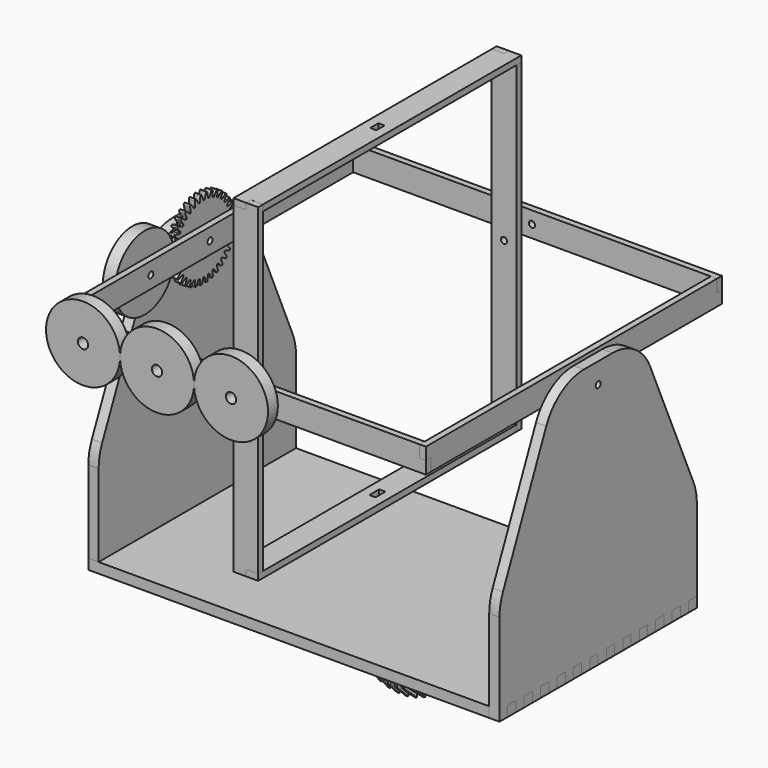
from build123d import *

# Parameters (mm, degrees)
F1_DEPTH  = 5
F2_R      = 1.5
F3_DEPTH  = 5
F4_R      = 1.5
F5_DEPTH  = 5
F6_R      = 1.5
F7_DEPTH  = 3
F8_R      = 1.5
F9_DEPTH  = 3
F10_R     = 1.5
F11_DEPTH = 3
F12_R     = 1.5
F13_DEPTH = 3
F14_R     = 1.5
F15_DEPTH = 3
F16_R     = 1.5
F17_DEPTH = 3
F18_W     = 3
F18_H     = 5
F19_DEPTH = 3
F20_R     = 1.5
F21_DEPTH = 3
F22_W     = 3
F22_H     = 6
F23_DEPTH = 3
F26_R     = 18
F26_R_2   = 2.5
F27_DEPTH = 6
F28_R     = 18
F28_R_2   = 2.5
F29_DEPTH = 6
F30_R     = 18
F30_R_2   = 2.5
F31_DEPTH = 6
F32_R     = 18
F32_R_2   = 2.5
F33_DEPTH = 6
F40_R     = 2.5
F41_DEPTH = 25


# Not quite as in the source:
# - a feature of the source that left no trace in its solid (it failed there, or was rolled back) is left out


with BuildPart() as f1:
    # F0 (on Top) → F1 (new body)
    with BuildSketch(Plane.XY):
        Polygon((100, 55), (100, 60), (-95, 60), (-95, 55), (-100, 55), (-100, 50), (-95, 50), (-95, 45), (-100, 45), (-100, 40), (-95, 40), (-95, 35), (-100, 35), (-100, 30), (-95, 30), (-95, 25), (-100, 25), (-100, 20), (-95, 20), (-95, 15), (-100, 15), (-100, 10), (-95, 10), (-95, 5), (-100, 5), (-100, 0), (-95, 0), (-95, -5), (-100, -5), (-100, -10), (-95, -10), (-95, -15), (-100, -15), (-100, -20), (-95, -20), (-95, -25), (-100, -25), (-100, -30), (-95, -30), (-95, -35), (-100, -35), (-100, -40), (-95, -40), (-95, -45), (-100, -45), (-100, -50), (-95, -50), (-95, -55), (-100, -55), (-100, -60), (95, -60), (95, -55), (100, -55), (100, -50), (95, -50), (95, -45), (100, -45), (100, -40), (95, -40), (95, -35), (100, -35), (100, -30), (95, -30), (95, -25), (100, -25), (100, -20), (95, -20), (95, -15), (100, -15), (100, -10), (95, -10), (95, -5), (100, -5), (100, 0), (95, 0), (95, 5), (100, 5), (100, 10), (95, 10), (95, 15), (100, 15), (100, 20), (95, 20), (95, 25), (100, 25), (100, 30), (95, 30), (95, 35), (100, 35), (100, 40), (95, 40), (95, 45), (100, 45), (100, 50), (95, 50), (95, 55), align=None)
    extrude(amount=F1_DEPTH)


with BuildPart() as f3:
    # F2 (on face) → F3 (new body)
    with BuildSketch(Plane.YZ.offset(100)):
        with BuildLine():
            Line((50, 0), (55, 0))
            Line((55, 0), (55, 5))
            Line((55, 5), (60, 5))
            Line((60, 5), (60, 44.7705385837))
            ThreePointArc((60, 44.7705385837), (59.4703732533, 49.8892134945), (57.9039333726, 54.7910094342))
            Line((57.9039333726, 54.7910094342), (31.5535440029, 115.0204708505))
            ThreePointArc((31.5535440029, 115.0204708505), (22.3333277558, 125.9226166057), (8.6496106304, 130))
            Line((8.6496106304, 130), (-8.6496106304, 130))
            ThreePointArc((-8.6496106304, 130), (-22.3333277558, 125.9226166057), (-31.5535440029, 115.0204708505))
            Line((-31.5535440029, 115.0204708505), (-57.9039333726, 54.7910094342))
            ThreePointArc((-57.9039333726, 54.7910094342), (-59.4703732533, 49.8892134945), (-60, 44.7705385837))
            Line((-60, 44.7705385837), (-60, 0))
            Line((-60, 0), (-55, 0))
            Line((-55, 0), (-55, 5))
            Line((-55, 5), (-50, 5))
            Line((-50, 5), (-50, 0))
            Line((-50, 0), (-45, 0))
            Line((-45, 0), (-45, 5))
            Line((-45, 5), (-40, 5))
            Line((-40, 5), (-40, 0))
            Line((-40, 0), (-35, 0))
            Line((-35, 0), (-35, 5))
            Line((-35, 5), (-30, 5))
            Line((-30, 5), (-30, 0))
            Line((-30, 0), (-25, 0))
            Line((-25, 0), (-25, 5))
            Line((-25, 5), (-20, 5))
            Line((-20, 5), (-20, 0))
            Line((-20, 0), (-15, 0))
            Line((-15, 0), (-15, 5))
            Line((-15, 5), (-10, 5))
            Line((-10, 5), (-10, 0))
            Line((-10, 0), (-5, 0))
            Line((-5, 0), (-5, 5))
            Line((-5, 5), (0, 5))
            Line((0, 5), (0, 0))
            Line((0, 0), (5, 0))
            Line((5, 0), (5, 5))
            Line((5, 5), (10, 5))
            Line((10, 5), (10, 0))
            Line((10, 0), (15, 0))
            Line((15, 0), (15, 5))
            Line((15, 5), (20, 5))
            Line((20, 5), (20, 0))
            Line((20, 0), (25, 0))
            Line((25, 0), (25, 5))
            Line((25, 5), (30, 5))
            Line((30, 5), (30, 0))
            Line((30, 0), (35, 0))
            Line((35, 0), (35, 5))
            Line((35, 5), (40, 5))
            Line((40, 5), (40, 0))
            Line((40, 0), (45, 0))
            Line((45, 0), (45, 5))
            Line((45, 5), (50, 5))
            Line((50, 5), (50, 0))
        make_face()
        with Locations((0, 120)):
            Circle(F2_R, mode=Mode.SUBTRACT)
    extrude(amount=-F3_DEPTH)


with BuildPart() as f5:
    # F4 (on face) → F5 (new body)
    with BuildSketch(Plane(origin=(-100, 0, 0), x_dir=(0, -1, 0), z_dir=(-1, 0, 0))):
        with BuildLine():
            Line((50, 0), (55, 0))
            Line((55, 0), (55, 5))
            Line((55, 5), (60, 5))
            Line((60, 5), (60, 45.0277700469))
            ThreePointArc((60, 45.0277700469), (59.4580269805, 50.2051164927), (57.8556067024, 55.1579843716))
            Line((57.8556067024, 55.1579843716), (31.2743152553, 115.1302143247))
            ThreePointArc((31.2743152553, 115.1302143247), (22.0522085049, 125.9553735128), (8.4187085529, 130))
            Line((8.4187085529, 130), (-8.9065918714, 130))
            ThreePointArc((-8.9065918714, 130), (-22.6250646146, 125.8998446308), (-31.8437077839, 114.9442804474))
            Line((-31.8437077839, 114.9442804474), (-57.9371159125, 54.7581734726))
            ThreePointArc((-57.9371159125, 54.7581734726), (-59.4788469685, 49.8918897851), (-60, 44.8138930252))
            Line((-60, 44.8138930252), (-60, 0))
            Line((-60, 0), (-55, 0))
            Line((-55, 0), (-55, 5))
            Line((-55, 5), (-50, 5))
            Line((-50, 5), (-50, 0))
            Line((-50, 0), (-45, 0))
            Line((-45, 0), (-45, 5))
            Line((-45, 5), (-40, 5))
            Line((-40, 5), (-40, 0))
            Line((-40, 0), (-35, 0))
            Line((-35, 0), (-35, 5))
            Line((-35, 5), (-30, 5))
            Line((-30, 5), (-30, 0))
            Line((-30, 0), (-25, 0))
            Line((-25, 0), (-25, 5))
            Line((-25, 5), (-20, 5))
            Line((-20, 5), (-20, 0))
            Line((-20, 0), (-15, 0))
            Line((-15, 0), (-15, 5))
            Line((-15, 5), (-10, 5))
            Line((-10, 5), (-10, 0))
            Line((-10, 0), (-5, 0))
            Line((-5, 0), (-5, 5))
            Line((-5, 5), (0, 5))
            Line((0, 5), (0, 0))
            Line((0, 0), (5, 0))
            Line((5, 0), (5, 5))
            Line((5, 5), (10, 5))
            Line((10, 5), (10, 0))
            Line((10, 0), (15, 0))
            Line((15, 0), (15, 5))
            Line((15, 5), (20, 5))
            Line((20, 5), (20, 0))
            Line((20, 0), (25, 0))
            Line((25, 0), (25, 5))
            Line((25, 5), (30, 5))
            Line((30, 5), (30, 0))
            Line((30, 0), (35, 0))
            Line((35, 0), (35, 5))
            Line((35, 5), (40, 5))
            Line((40, 5), (40, 0))
            Line((40, 0), (45, 0))
            Line((45, 0), (45, 5))
            Line((45, 5), (50, 5))
            Line((50, 5), (50, 0))
        make_face()
        with Locations((-0.2439416593, 120)):
            Circle(F4_R, mode=Mode.SUBTRACT)
    extrude(amount=-F5_DEPTH)


with BuildPart() as f7:
    # F6 (on face) → F7 (new body)
    with BuildSketch(Plane.YZ.offset(-95)):
        with BuildLine():
            ThreePointArc((-0.9074454432, 138.9766193212), (-1.1059043827, 139.2442584986), (-1.4284580066, 139.3277799904))
            ThreePointArc((-1.4284580066, 139.3277799904), (-1.44687975, 139.326177143), (-1.4652999573, 139.3245567374))
            ThreePointArc((-1.4652999573, 139.3245567374), (-1.7684499121, 139.1862932757), (-1.9174187589, 138.8882581056))
            Line((-1.9174187589, 138.8882581056), (-2.2042135214, 136.5840744477))
            ThreePointArc((-2.2042135214, 136.5840744477), (-2.3348708966, 136.3046577179), (-2.6046356928, 136.1550849487))
            ThreePointArc((-2.6046356928, 136.1550849487), (-2.9092885812, 136.2033723819), (-3.1276325025, 136.4212507668))
            Line((-3.1276325025, 136.4212507668), (-4.1852086494, 138.4883855613))
            ThreePointArc((-4.1852086494, 138.4883855613), (-4.427127607, 138.7174966651), (-4.7592842715, 138.7437384288))
            ThreePointArc((-4.7592842715, 138.7437384288), (-4.7771478157, 138.73896103), (-4.7950067982, 138.7341666066))
            ThreePointArc((-4.7950067982, 138.7341666066), (-5.0695420259, 138.5453622404), (-5.164494437, 138.2259867254))
            Line((-5.164494437, 138.2259867254), (-5.0468148493, 135.9070074068))
            ThreePointArc((-5.0468148493, 135.9070074068), (-5.1269670395, 135.6091472299), (-5.3666604635, 135.415002642))
            ThreePointArc((-5.3666604635, 135.415002642), (-5.6750700147, 135.4096540616), (-5.9279309858, 135.5863073602))
            Line((-5.9279309858, 135.5863073602), (-7.3283943647, 137.4383915618))
            ThreePointArc((-7.3283943647, 137.4383915618), (-7.6064227554, 137.6220131669), (-7.9380900483, 137.5901778597))
            ThreePointArc((-7.9380900483, 137.5901778597), (-7.9548526185, 137.5823710685), (-7.97160774, 137.5745483034))
            ThreePointArc((-7.97160774, 137.5745483034), (-8.2091866266, 137.3409397577), (-8.247237521, 137.0099279613))
            Line((-8.247237521, 137.0099279613), (-7.728659218, 134.7466139953))
            ThreePointArc((-7.728659218, 134.7466139953), (-7.7558708394, 134.439360702), (-7.9582099279, 134.2065432803))
            ThreePointArc((-7.9582099279, 134.2065432803), (-8.2610052737, 134.1477212004), (-8.5407002418, 134.2777818916))
            Line((-8.5407002418, 134.2777818916), (-10.2414984817, 135.8585408589))
            ThreePointArc((-10.2414984817, 135.8585408589), (-10.5471885535, 135.9910937158), (-10.8682889319, 135.9021486375))
            ThreePointArc((-10.8682889319, 135.9021486375), (-10.883441206, 135.8915496592), (-10.8985833706, 135.8809362432))
            ThreePointArc((-10.8985833706, 135.8809362432), (-11.0919872018, 135.6096215955), (-11.0719804224, 135.2770311436))
            Line((-11.0719804224, 135.2770311436), (-10.1682601434, 133.1381521796))
            ThreePointArc((-10.1682601434, 133.1381521796), (-10.1417043847, 132.8308415058), (-10.3005411667, 132.5664252899))
            ThreePointArc((-10.3005411667, 132.5664252899), (-10.5885220239, 132.4559169895), (-10.886552599, 132.5354332451))
            Line((-10.886552599, 132.5354332451), (-12.8360078059, 133.7968364168))
            ThreePointArc((-12.8360078059, 133.7968364168), (-13.1600713207, 133.8742929741), (-13.4608483121, 133.7309406758))
            ThreePointArc((-13.4608483121, 133.7309406758), (-13.4739298958, 133.717871555), (-13.4869990165, 133.7047899713))
            ThreePointArc((-13.4869990165, 133.7047899713), (-13.6303513148, 133.40401298), (-13.5528947575, 133.0799494651))
            Line((-13.5528947575, 133.0799494651), (-12.2914915858, 131.1304942582))
            ThreePointArc((-12.2914915858, 131.1304942582), (-12.2119753303, 130.8324636832), (-12.3224836306, 130.5444828259))
            ThreePointArc((-12.3224836306, 130.5444828259), (-12.5868998465, 130.3856460439), (-12.8942105204, 130.4122018027))
            Line((-12.8942105204, 130.4122018027), (-15.0330894843, 131.3159220817))
            ThreePointArc((-15.0330894843, 131.3159220817), (-15.3656799363, 131.335928861), (-15.6369945839, 131.1425250298))
            ThreePointArc((-15.6369945839, 131.1425250298), (-15.647608, 131.1273828652), (-15.6582069782, 131.1122305911))
            ThreePointArc((-15.6582069782, 131.1122305911), (-15.7471520566, 130.7911302128), (-15.6145991996, 130.4854401409))
            Line((-15.6145991996, 130.4854401409), (-14.0338402323, 128.7846419011))
            ThreePointArc((-14.0338402323, 128.7846419011), (-13.9037795411, 128.504946933), (-13.962601621, 128.2021515871))
            ThreePointArc((-13.962601621, 128.2021515871), (-14.1954190427, 127.9998124987), (-14.502672336, 127.9726008773))
            Line((-14.502672336, 127.9726008773), (-16.7659863021, 128.4911791803))
            ThreePointArc((-16.7659863021, 128.4911791803), (-17.0969980985, 128.4531282858), (-17.3306066441, 128.2155493993))
            ThreePointArc((-17.3306066441, 128.2155493993), (-17.3384294093, 128.1987942778), (-17.3462362005, 128.1820317075))
            ThreePointArc((-17.3462362005, 128.1820317075), (-17.3780715077, 127.8503644147), (-17.1944499025, 127.5723360239))
            Line((-17.1944499025, 127.5723360239), (-15.342365701, 126.171872645))
            ThreePointArc((-15.342365701, 126.171872645), (-15.1657124024, 125.919011674), (-15.1710609827, 125.6106021228))
            ThreePointArc((-15.1710609827, 125.6106021228), (-15.3652055707, 125.3709086988), (-15.6630657476, 125.2907565086))
            Line((-15.6630657476, 125.2907565086), (-17.9820450661, 125.4084360962))
            ThreePointArc((-17.9820450661, 125.4084360962), (-18.3014205811, 125.3134836851), (-18.4902249473, 125.0389484574))
            ThreePointArc((-18.4902249473, 125.0389484574), (-18.4950193708, 125.021089475), (-18.4997967695, 125.0032259308))
            ThreePointArc((-18.4997967695, 125.0032259308), (-18.4735550058, 124.6710692663), (-18.2444439021, 124.4291503086))
            Line((-18.2444439021, 124.4291503086), (-16.1773091075, 123.3715741617))
            ThreePointArc((-16.1773091075, 123.3715741617), (-15.9594307227, 123.1532302404), (-15.9111432895, 122.8485773521))
            ThreePointArc((-15.9111432895, 122.8485773521), (-16.0607160587, 122.5788125559), (-16.3401327884, 122.4481551806))
            Line((-16.3401327884, 122.4481551806), (-18.6443164463, 122.1613604182))
            ThreePointArc((-18.6443164463, 122.1613604182), (-18.9423516165, 122.0123915714), (-19.0806150781, 121.7092416166))
            ThreePointArc((-19.0806150781, 121.7092416166), (-19.0822354837, 121.6908214093), (-19.0838383312, 121.6723996659))
            ThreePointArc((-19.0838383312, 121.6723996659), (-19.0003168394, 121.3498460419), (-18.7326776619, 121.1513871025))
            Line((-18.7326776619, 121.1513871025), (-16.5133011191, 120.4688321037))
            ThreePointArc((-16.5133011191, 120.4688321037), (-16.2608177724, 120.2916395016), (-16.160361515, 120))
            ThreePointArc((-16.160361515, 120), (-16.2608177724, 119.7083604984), (-16.5133011191, 119.5311678963))
            Line((-16.5133011191, 119.5311678963), (-18.7326776619, 118.8486128975))
            ThreePointArc((-18.7326776619, 118.8486128975), (-19.0003168394, 118.6501539581), (-19.0838383312, 118.3276003341))
            ThreePointArc((-19.0838383312, 118.3276003341), (-19.0822354837, 118.3091785907), (-19.0806150781, 118.2907583834))
            ThreePointArc((-19.0806150781, 118.2907583834), (-18.9423516165, 117.9876084286), (-18.6443164463, 117.8386395818))
            Line((-18.6443164463, 117.8386395818), (-16.3401327884, 117.5518448194))
            ThreePointArc((-16.3401327884, 117.5518448194), (-16.0607160587, 117.4211874442), (-15.9111432895, 117.1514226479))
            ThreePointArc((-15.9111432895, 117.1514226479), (-15.9594307227, 116.8467697596), (-16.1773091075, 116.6284258383))
            Line((-16.1773091075, 116.6284258383), (-18.2444439021, 115.5708496914))
            ThreePointArc((-18.2444439021, 115.5708496914), (-18.4735550058, 115.3289307337), (-18.4997967695, 114.9967740692))
            ThreePointArc((-18.4997967695, 114.9967740692), (-18.4950193708, 114.978910525), (-18.4902249473, 114.9610515426))
            ThreePointArc((-18.4902249473, 114.9610515426), (-18.3014205811, 114.6865163149), (-17.9820450661, 114.5915639038))
            Line((-17.9820450661, 114.5915639038), (-15.6630657476, 114.7092434914))
            ThreePointArc((-15.6630657476, 114.7092434914), (-15.3652055707, 114.6290913012), (-15.1710609827, 114.3893978772))
            ThreePointArc((-15.1710609827, 114.3893978772), (-15.1657124024, 114.080988326), (-15.342365701, 113.828127355))
            Line((-15.342365701, 113.828127355), (-17.1944499025, 112.4276639761))
            ThreePointArc((-17.1944499025, 112.4276639761), (-17.3780715077, 112.1496355853), (-17.3462362005, 111.8179682925))
            ThreePointArc((-17.3462362005, 111.8179682925), (-17.3384294093, 111.8012057222), (-17.3306066441, 111.7844506007))
            ThreePointArc((-17.3306066441, 111.7844506007), (-17.0969980985, 111.5468717142), (-16.7659863021, 111.5088208197))
            Line((-16.7659863021, 111.5088208197), (-14.502672336, 112.0273991227))
            ThreePointArc((-14.502672336, 112.0273991227), (-14.1954190427, 112.0001875013), (-13.962601621, 111.7978484129))
            ThreePointArc((-13.962601621, 111.7978484129), (-13.9037795411, 111.495053067), (-14.0338402323, 111.2153580989))
            Line((-14.0338402323, 111.2153580989), (-15.6145991996, 109.5145598591))
            ThreePointArc((-15.6145991996, 109.5145598591), (-15.7471520566, 109.2088697872), (-15.6582069782, 108.8877694089))
            ThreePointArc((-15.6582069782, 108.8877694089), (-15.647608, 108.8726171348), (-15.6369945839, 108.8574749702))
            ThreePointArc((-15.6369945839, 108.8574749702), (-15.3656799363, 108.664071139), (-15.0330894843, 108.6840779183))
            Line((-15.0330894843, 108.6840779183), (-12.8942105204, 109.5877981973))
            ThreePointArc((-12.8942105204, 109.5877981973), (-12.5868998465, 109.6143539561), (-12.3224836306, 109.4555171741))
            ThreePointArc((-12.3224836306, 109.4555171741), (-12.2119753303, 109.1675363168), (-12.2914915858, 108.8695057418))
            Line((-12.2914915858, 108.8695057418), (-13.5528947575, 106.9200505349))
            ThreePointArc((-13.5528947575, 106.9200505349), (-13.6303513148, 106.59598702), (-13.4869990165, 106.2952100287))
            ThreePointArc((-13.4869990165, 106.2952100287), (-13.4739298958, 106.282128445), (-13.4608483121, 106.2690593242))
            ThreePointArc((-13.4608483121, 106.2690593242), (-13.1600713207, 106.1257070259), (-12.8360078059, 106.2031635832))
            Line((-12.8360078059, 106.2031635832), (-10.886552599, 107.4645667549))
            ThreePointArc((-10.886552599, 107.4645667549), (-10.5885220239, 107.5440830105), (-10.3005411667, 107.4335747102))
            ThreePointArc((-10.3005411667, 107.4335747102), (-10.1417043847, 107.1691584942), (-10.1682601434, 106.8618478204))
            Line((-10.1682601434, 106.8618478204), (-11.0719804224, 104.7229688564))
            ThreePointArc((-11.0719804224, 104.7229688564), (-11.0919872018, 104.3903784045), (-10.8985833706, 104.1190637568))
            ThreePointArc((-10.8985833706, 104.1190637568), (-10.883441206, 104.1084503408), (-10.8682889319, 104.0978513625))
            ThreePointArc((-10.8682889319, 104.0978513625), (-10.5471885535, 104.0089062842), (-10.2414984817, 104.1414591411))
            Line((-10.2414984817, 104.1414591411), (-8.5407002418, 105.7222181084))
            ThreePointArc((-8.5407002418, 105.7222181084), (-8.2610052737, 105.8522787996), (-7.9582099279, 105.7934567197))
            ThreePointArc((-7.9582099279, 105.7934567197), (-7.7558708394, 105.560639298), (-7.728659218, 105.2533860047))
            Line((-7.728659218, 105.2533860047), (-8.247237521, 102.9900720387))
            ThreePointArc((-8.247237521, 102.9900720387), (-8.2091866266, 102.6590602423), (-7.97160774, 102.4254516966))
            ThreePointArc((-7.97160774, 102.4254516966), (-7.9548526185, 102.4176289315), (-7.9380900483, 102.4098221403))
            ThreePointArc((-7.9380900483, 102.4098221403), (-7.6064227554, 102.3779868331), (-7.3283943647, 102.5616084382))
            Line((-7.3283943647, 102.5616084382), (-5.9279309858, 104.4136926398))
            ThreePointArc((-5.9279309858, 104.4136926398), (-5.6750700147, 104.5903459384), (-5.3666604636, 104.5849973581))
            ThreePointArc((-5.3666604636, 104.5849973581), (-5.1269670395, 104.3908527701), (-5.0468148493, 104.0929925932))
            Line((-5.0468148493, 104.0929925932), (-5.164494437, 101.7740132746))
            ThreePointArc((-5.164494437, 101.7740132746), (-5.0695420259, 101.4546377596), (-4.7950067982, 101.2658333934))
            ThreePointArc((-4.7950067982, 101.2658333934), (-4.7771478157, 101.26103897), (-4.7592842715, 101.2562615712))
            ThreePointArc((-4.7592842715, 101.2562615712), (-4.427127607, 101.2825033349), (-4.1852086494, 101.5116144387))
            Line((-4.1852086494, 101.5116144387), (-3.1276325025, 103.5787492332))
            ThreePointArc((-3.1276325025, 103.5787492332), (-2.9092885812, 103.7966276181), (-2.6046356928, 103.8449150513))
            ThreePointArc((-2.6046356928, 103.8449150513), (-2.3348708966, 103.6953422821), (-2.2042135214, 103.4159255523))
            Line((-2.2042135214, 103.4159255523), (-1.9174187589, 101.1117418944))
            ThreePointArc((-1.9174187589, 101.1117418944), (-1.7684499121, 100.8137067243), (-1.4652999573, 100.6754432626))
            ThreePointArc((-1.4652999573, 100.6754432626), (-1.44687975, 100.673822857), (-1.4284580066, 100.6722200096))
            ThreePointArc((-1.4284580066, 100.6722200096), (-1.1059043827, 100.7557415014), (-0.9074454432, 101.0233806788))
            Line((-0.9074454432, 101.0233806788), (-0.2248904444, 103.2427572216))
            ThreePointArc((-0.2248904444, 103.2427572216), (-0.0476978424, 103.4952405683), (0.2439416592, 103.5956968258))
            ThreePointArc((0.2439416592, 103.5956968258), (0.5355811609, 103.4952405683), (0.7127737629, 103.2427572216))
            Line((0.7127737629, 103.2427572216), (1.3953287617, 101.0233806788))
            ThreePointArc((1.3953287617, 101.0233806788), (1.5937877012, 100.7557415014), (1.9163413251, 100.6722200096))
            ThreePointArc((1.9163413251, 100.6722200096), (1.9347630686, 100.673822857), (1.9531832758, 100.6754432626))
            ThreePointArc((1.9531832758, 100.6754432626), (2.2563332306, 100.8137067243), (2.4053020774, 101.1117418944))
            Line((2.4053020774, 101.1117418944), (2.6920968399, 103.4159255523))
            ThreePointArc((2.6920968399, 103.4159255523), (2.8227542151, 103.6953422821), (3.0925190113, 103.8449150513))
            ThreePointArc((3.0925190113, 103.8449150513), (3.3971718997, 103.7966276181), (3.615515821, 103.5787492332))
            Line((3.615515821, 103.5787492332), (4.6730919679, 101.5116144387))
            ThreePointArc((4.6730919679, 101.5116144387), (4.9150109255, 101.2825033349), (5.24716759, 101.2562615712))
            ThreePointArc((5.24716759, 101.2562615712), (5.2650311342, 101.26103897), (5.2828901167, 101.2658333934))
            ThreePointArc((5.2828901167, 101.2658333934), (5.5574253444, 101.4546377596), (5.6523777555, 101.7740132746))
            Line((5.6523777555, 101.7740132746), (5.5346981678, 104.0929925932))
            ThreePointArc((5.5346981678, 104.0929925932), (5.614850358, 104.3908527701), (5.8545437821, 104.584997358))
            ThreePointArc((5.8545437821, 104.584997358), (6.1629533332, 104.5903459384), (6.4158143043, 104.4136926398))
            Line((6.4158143043, 104.4136926398), (7.8162776832, 102.5616084382))
            ThreePointArc((7.8162776832, 102.5616084382), (8.0943060739, 102.3779868331), (8.4259733668, 102.4098221403))
            ThreePointArc((8.4259733668, 102.4098221403), (8.442735937, 102.4176289315), (8.4594910585, 102.4254516966))
            ThreePointArc((8.4594910585, 102.4254516966), (8.6970699451, 102.6590602423), (8.7351208395, 102.9900720387))
            Line((8.7351208395, 102.9900720387), (8.2165425365, 105.2533860047))
            ThreePointArc((8.2165425365, 105.2533860047), (8.2437541579, 105.560639298), (8.4460932464, 105.7934567197))
            ThreePointArc((8.4460932464, 105.7934567197), (8.7488885922, 105.8522787996), (9.0285835603, 105.7222181084))
            Line((9.0285835603, 105.7222181084), (10.7293818002, 104.1414591411))
            ThreePointArc((10.7293818002, 104.1414591411), (11.0350718721, 104.0089062842), (11.3561722504, 104.0978513625))
            ThreePointArc((11.3561722504, 104.0978513625), (11.3713245245, 104.1084503408), (11.3864666891, 104.1190637568))
            ThreePointArc((11.3864666891, 104.1190637568), (11.5798705203, 104.3903784045), (11.5598637409, 104.7229688564))
            Line((11.5598637409, 104.7229688564), (10.6561434619, 106.8618478204))
            ThreePointArc((10.6561434619, 106.8618478204), (10.6295877032, 107.1691584942), (10.7884244852, 107.4335747101))
            ThreePointArc((10.7884244852, 107.4335747101), (11.0764053424, 107.5440830105), (11.3744359175, 107.4645667549))
            Line((11.3744359175, 107.4645667549), (13.3238911244, 106.2031635832))
            ThreePointArc((13.3238911244, 106.2031635832), (13.6479546392, 106.1257070259), (13.9487316306, 106.2690593242))
            ThreePointArc((13.9487316306, 106.2690593242), (13.9618132143, 106.282128445), (13.9748823351, 106.2952100287))
            ThreePointArc((13.9748823351, 106.2952100287), (14.1182346333, 106.59598702), (14.040778076, 106.9200505349))
            Line((14.040778076, 106.9200505349), (12.7793749043, 108.8695057418))
            ThreePointArc((12.7793749043, 108.8695057418), (12.6998586488, 109.1675363168), (12.8103669491, 109.4555171741))
            ThreePointArc((12.8103669491, 109.4555171741), (13.074783165, 109.6143539561), (13.3820938389, 109.5877981973))
            Line((13.3820938389, 109.5877981973), (15.5209728028, 108.6840779183))
            ThreePointArc((15.5209728028, 108.6840779183), (15.8535632548, 108.664071139), (16.1248779024, 108.8574749702))
            ThreePointArc((16.1248779024, 108.8574749702), (16.1354913185, 108.8726171348), (16.1460902968, 108.8877694089))
            ThreePointArc((16.1460902968, 108.8877694089), (16.2350353751, 109.2088697872), (16.1024825181, 109.5145598591))
            Line((16.1024825181, 109.5145598591), (14.5217235509, 111.2153580989))
            ThreePointArc((14.5217235509, 111.2153580989), (14.3916628596, 111.495053067), (14.4504849395, 111.7978484129))
            ThreePointArc((14.4504849395, 111.7978484129), (14.6833023613, 112.0001875013), (14.9905556545, 112.0273991227))
            Line((14.9905556545, 112.0273991227), (17.2538696206, 111.5088208197))
            ThreePointArc((17.2538696206, 111.5088208197), (17.584881417, 111.5468717142), (17.8184899626, 111.7844506007))
            ThreePointArc((17.8184899626, 111.7844506007), (17.8263127278, 111.8012057222), (17.834119519, 111.8179682925))
            ThreePointArc((17.834119519, 111.8179682925), (17.8659548262, 112.1496355853), (17.682333221, 112.4276639761))
            Line((17.682333221, 112.4276639761), (15.8302490195, 113.828127355))
            ThreePointArc((15.8302490195, 113.828127355), (15.6535957209, 114.080988326), (15.6589443012, 114.3893978772))
            ThreePointArc((15.6589443012, 114.3893978772), (15.8530888892, 114.6290913012), (16.1509490661, 114.7092434914))
            Line((16.1509490661, 114.7092434914), (18.4699283846, 114.5915639038))
            ThreePointArc((18.4699283846, 114.5915639038), (18.7893038996, 114.6865163149), (18.9781082658, 114.9610515426))
            ThreePointArc((18.9781082658, 114.9610515426), (18.9829026893, 114.978910525), (18.987680088, 114.9967740692))
            ThreePointArc((18.987680088, 114.9967740692), (18.9614383244, 115.3289307337), (18.7323272206, 115.5708496914))
            Line((18.7323272206, 115.5708496914), (16.6651924261, 116.6284258383))
            ThreePointArc((16.6651924261, 116.6284258383), (16.4473140412, 116.8467697596), (16.399026608, 117.1514226479))
            ThreePointArc((16.399026608, 117.1514226479), (16.5485993772, 117.4211874441), (16.8280161069, 117.5518448194))
            Line((16.8280161069, 117.5518448194), (19.1321997648, 117.8386395818))
            ThreePointArc((19.1321997648, 117.8386395818), (19.430234935, 117.9876084286), (19.5684983966, 118.2907583834))
            ThreePointArc((19.5684983966, 118.2907583834), (19.5701188022, 118.3091785907), (19.5717216497, 118.3276003341))
            ThreePointArc((19.5717216497, 118.3276003341), (19.4882001579, 118.6501539581), (19.2205609804, 118.8486128975))
            Line((19.2205609804, 118.8486128975), (17.0011844376, 119.5311678963))
            ThreePointArc((17.0011844376, 119.5311678963), (16.7487010909, 119.7083604984), (16.6482448335, 120))
            ThreePointArc((16.6482448335, 120), (16.7487010909, 120.2916395016), (17.0011844376, 120.4688321037))
            Line((17.0011844376, 120.4688321037), (19.2205609804, 121.1513871025))
            ThreePointArc((19.2205609804, 121.1513871025), (19.4882001579, 121.3498460419), (19.5717216497, 121.6723996659))
            ThreePointArc((19.5717216497, 121.6723996659), (19.5701188022, 121.6908214093), (19.5684983966, 121.7092416166))
            ThreePointArc((19.5684983966, 121.7092416166), (19.430234935, 122.0123915714), (19.1321997648, 122.1613604182))
            Line((19.1321997648, 122.1613604182), (16.8280161069, 122.4481551806))
            ThreePointArc((16.8280161069, 122.4481551806), (16.5485993772, 122.5788125558), (16.399026608, 122.8485773521))
            ThreePointArc((16.399026608, 122.8485773521), (16.4473140412, 123.1532302404), (16.6651924261, 123.3715741617))
            Line((16.6651924261, 123.3715741617), (18.7323272206, 124.4291503086))
            ThreePointArc((18.7323272206, 124.4291503086), (18.9614383244, 124.6710692663), (18.987680088, 125.0032259308))
            ThreePointArc((18.987680088, 125.0032259308), (18.9829026893, 125.021089475), (18.9781082658, 125.0389484574))
            ThreePointArc((18.9781082658, 125.0389484574), (18.7893038996, 125.3134836851), (18.4699283846, 125.4084360962))
            Line((18.4699283846, 125.4084360962), (16.1509490661, 125.2907565086))
            ThreePointArc((16.1509490661, 125.2907565086), (15.8530888892, 125.3709086988), (15.6589443012, 125.6106021228))
            ThreePointArc((15.6589443012, 125.6106021228), (15.6535957209, 125.919011674), (15.8302490195, 126.171872645))
            Line((15.8302490195, 126.171872645), (17.682333221, 127.5723360239))
            ThreePointArc((17.682333221, 127.5723360239), (17.8659548262, 127.8503644147), (17.834119519, 128.1820317075))
            ThreePointArc((17.834119519, 128.1820317075), (17.8263127278, 128.1987942778), (17.8184899626, 128.2155493993))
            ThreePointArc((17.8184899626, 128.2155493993), (17.584881417, 128.4531282858), (17.2538696206, 128.4911791803))
            Line((17.2538696206, 128.4911791803), (14.9905556545, 127.9726008773))
            ThreePointArc((14.9905556545, 127.9726008773), (14.6833023613, 127.9998124987), (14.4504849395, 128.2021515871))
            ThreePointArc((14.4504849395, 128.2021515871), (14.3916628596, 128.504946933), (14.5217235509, 128.7846419011))
            Line((14.5217235509, 128.7846419011), (16.1024825181, 130.4854401409))
            ThreePointArc((16.1024825181, 130.4854401409), (16.2350353751, 130.7911302128), (16.1460902968, 131.1122305911))
            ThreePointArc((16.1460902968, 131.1122305911), (16.1354913185, 131.1273828652), (16.1248779024, 131.1425250298))
            ThreePointArc((16.1248779024, 131.1425250298), (15.8535632548, 131.335928861), (15.5209728028, 131.3159220817))
            Line((15.5209728028, 131.3159220817), (13.3820938389, 130.4122018027))
            ThreePointArc((13.3820938389, 130.4122018027), (13.0747831651, 130.3856460439), (12.8103669491, 130.5444828259))
            ThreePointArc((12.8103669491, 130.5444828259), (12.6998586488, 130.8324636832), (12.7793749043, 131.1304942582))
            Line((12.7793749043, 131.1304942582), (14.040778076, 133.0799494651))
            ThreePointArc((14.040778076, 133.0799494651), (14.1182346333, 133.40401298), (13.9748823351, 133.7047899713))
            ThreePointArc((13.9748823351, 133.7047899713), (13.9618132143, 133.717871555), (13.9487316306, 133.7309406758))
            ThreePointArc((13.9487316306, 133.7309406758), (13.6479546392, 133.8742929741), (13.3238911244, 133.7968364168))
            Line((13.3238911244, 133.7968364168), (11.3744359175, 132.5354332451))
            ThreePointArc((11.3744359175, 132.5354332451), (11.0764053424, 132.4559169895), (10.7884244852, 132.5664252898))
            ThreePointArc((10.7884244852, 132.5664252898), (10.6295877032, 132.8308415058), (10.6561434619, 133.1381521796))
            Line((10.6561434619, 133.1381521796), (11.5598637409, 135.2770311436))
            ThreePointArc((11.5598637409, 135.2770311436), (11.5798705203, 135.6096215955), (11.3864666891, 135.8809362432))
            ThreePointArc((11.3864666891, 135.8809362432), (11.3713245245, 135.8915496592), (11.3561722504, 135.9021486375))
            ThreePointArc((11.3561722504, 135.9021486375), (11.0350718721, 135.9910937158), (10.7293818002, 135.8585408589))
            Line((10.7293818002, 135.8585408589), (9.0285835603, 134.2777818916))
            ThreePointArc((9.0285835603, 134.2777818916), (8.7488885923, 134.1477212004), (8.4460932464, 134.2065432803))
            ThreePointArc((8.4460932464, 134.2065432803), (8.2437541579, 134.439360702), (8.2165425365, 134.7466139953))
            Line((8.2165425365, 134.7466139953), (8.7351208395, 137.0099279613))
            ThreePointArc((8.7351208395, 137.0099279613), (8.6970699451, 137.3409397577), (8.4594910585, 137.5745483034))
            ThreePointArc((8.4594910585, 137.5745483034), (8.442735937, 137.5823710685), (8.4259733668, 137.5901778597))
            ThreePointArc((8.4259733668, 137.5901778597), (8.0943060739, 137.6220131669), (7.8162776832, 137.4383915618))
            Line((7.8162776832, 137.4383915618), (6.4158143043, 135.5863073602))
            ThreePointArc((6.4158143043, 135.5863073602), (6.1629533332, 135.4096540616), (5.8545437821, 135.4150026419))
            ThreePointArc((5.8545437821, 135.4150026419), (5.614850358, 135.6091472299), (5.5346981678, 135.9070074068))
            Line((5.5346981678, 135.9070074068), (5.6523777555, 138.2259867254))
            ThreePointArc((5.6523777555, 138.2259867254), (5.5574253444, 138.5453622404), (5.2828901167, 138.7341666066))
            ThreePointArc((5.2828901167, 138.7341666066), (5.2650311342, 138.73896103), (5.24716759, 138.7437384288))
            ThreePointArc((5.24716759, 138.7437384288), (4.9150109255, 138.7174966651), (4.6730919679, 138.4883855613))
            Line((4.6730919679, 138.4883855613), (3.615515821, 136.4212507668))
            ThreePointArc((3.615515821, 136.4212507668), (3.3971718997, 136.2033723819), (3.0925190114, 136.1550849487))
            ThreePointArc((3.0925190114, 136.1550849487), (2.8227542151, 136.3046577179), (2.6920968399, 136.5840744477))
            Line((2.6920968399, 136.5840744477), (2.4053020774, 138.8882581056))
            ThreePointArc((2.4053020774, 138.8882581056), (2.2563332306, 139.1862932757), (1.9531832758, 139.3245567374))
            ThreePointArc((1.9531832758, 139.3245567374), (1.9347630686, 139.326177143), (1.9163413251, 139.3277799904))
            ThreePointArc((1.9163413251, 139.3277799904), (1.5937877012, 139.2442584986), (1.3953287617, 138.9766193212))
            Line((1.3953287617, 138.9766193212), (0.7127737629, 136.7572427784))
            ThreePointArc((0.7127737629, 136.7572427784), (0.5355811609, 136.5047594317), (0.2439416593, 136.4043031742))
            ThreePointArc((0.2439416593, 136.4043031742), (-0.0476978424, 136.5047594317), (-0.2248904444, 136.7572427784))
            Line((-0.2248904444, 136.7572427784), (-0.9074454432, 138.9766193212))
        make_face()
        with BuildLine():
            ThreePointArc((-10.2852554216, 107.4207006941), (-10.2928339664, 107.4272140806), (-10.3005411667, 107.4335747102))
            ThreePointArc((-10.3005411667, 107.4335747102), (-10.3081435053, 107.440060309), (-10.3158739393, 107.446392681))
            Line((-10.3158739393, 107.446392681), (-10.3002843799, 107.4338807368))
            Line((-10.3002843799, 107.4338807368), (-10.2852554216, 107.4207006941))
        make_face(mode=Mode.SUBTRACT)
        with BuildLine():
            ThreePointArc((-12.3096656598, 109.4401844015), (-12.3159980317, 109.4479148355), (-12.3224836306, 109.4555171741))
            ThreePointArc((-12.3224836306, 109.4555171741), (-12.3288442602, 109.4632243744), (-12.3353576467, 109.4708029192))
            Line((-12.3353576467, 109.4708029192), (-12.322177604, 109.4557739609))
            Line((-12.322177604, 109.4557739609), (-12.3096656598, 109.4401844015))
        make_face(mode=Mode.SUBTRACT)
        with BuildLine():
            ThreePointArc((-5.3478933889, 104.5781277729), (-5.3572426009, 104.5816563391), (-5.3666604636, 104.5849973581))
            ThreePointArc((-5.3666604636, 104.5849973581), (-5.3760225305, 104.5884916745), (-5.3854525611, 104.5917981936))
            Line((-5.3854525611, 104.5917981936), (-5.3665238301, 104.5853727553))
            Line((-5.3665238301, 104.5853727553), (-5.3478933889, 104.5781277729))
        make_face(mode=Mode.SUBTRACT)
        with BuildLine():
            ThreePointArc((-2.5849608413, 103.8414086988), (-2.5947807468, 103.8432601846), (-2.6046356928, 103.8449150513))
            ThreePointArc((-2.6046356928, 103.8449150513), (-2.6144623106, 103.8467305753), (-2.6243232489, 103.8483493533))
            Line((-2.6243232489, 103.8483493533), (-2.6045663222, 103.8453084715))
            Line((-2.6045663222, 103.8453084715), (-2.5849608413, 103.8414086988))
        make_face(mode=Mode.SUBTRACT)
        with BuildLine():
            ThreePointArc((-7.9409208582, 105.7834326307), (-7.9495153055, 105.7885310637), (-7.9582099279, 105.7934567197))
            ThreePointArc((-7.9582099279, 105.7934567197), (-7.9668229823, 105.7985236555), (-7.9755355785, 105.8034174488))
            Line((-7.9755355785, 105.8034174488), (-7.9580101832, 105.7938026877))
            Line((-7.9580101832, 105.7938026877), (-7.9409208582, 105.7834326307))
        make_face(mode=Mode.SUBTRACT)
        with BuildLine():
            ThreePointArc((-15.1642601472, 114.3706057797), (-15.1675666662, 114.3800358103), (-15.1710609827, 114.3893978772))
            ThreePointArc((-15.1710609827, 114.3893978772), (-15.1744020016, 114.3988157399), (-15.1779305679, 114.4081649519))
            Line((-15.1779305679, 114.4081649519), (-15.1706855855, 114.3895345106))
            Line((-15.1706855855, 114.3895345106), (-15.1642601472, 114.3706057797))
        make_face(mode=Mode.SUBTRACT)
        with BuildLine():
            ThreePointArc((-13.952640892, 111.7805227623), (-13.9575346852, 111.7892353585), (-13.962601621, 111.7978484129))
            ThreePointArc((-13.962601621, 111.7978484129), (-13.967527277, 111.8065430352), (-13.9726257101, 111.8151374826))
            Line((-13.9726257101, 111.8151374826), (-13.9622556531, 111.7980481576))
            Line((-13.9622556531, 111.7980481576), (-13.952640892, 111.7805227623))
        make_face(mode=Mode.SUBTRACT)
        with BuildLine():
            ThreePointArc((-15.9077089874, 117.1317350919), (-15.9093277654, 117.1415960301), (-15.9111432895, 117.1514226479))
            ThreePointArc((-15.9111432895, 117.1514226479), (-15.9127981561, 117.1612775939), (-15.9146496419, 117.1710974995))
            Line((-15.9146496419, 117.1710974995), (-15.9107498693, 117.1514920185))
            Line((-15.9107498693, 117.1514920185), (-15.9077089874, 117.1317350919))
        make_face(mode=Mode.SUBTRACT)
        with BuildLine():
            ThreePointArc((-16.1603980959, 119.9800151819), (-16.160279947, 119.9900074082), (-16.160361515, 120))
            ThreePointArc((-16.160361515, 120), (-16.160279947, 120.0099925918), (-16.1603980959, 120.0199848181))
            Line((-16.1603980959, 120.0199848181), (-16.1599620256, 120))
            Line((-16.1599620256, 120), (-16.1603980959, 119.9800151819))
        make_face(mode=Mode.SUBTRACT)
        with Locations((0.2439416593, 120)):
            Circle(F6_R, mode=Mode.SUBTRACT)
        with BuildLine():
            ThreePointArc((0.2639264773, 103.5956602449), (0.2539342511, 103.5957783937), (0.2439416592, 103.5956968258))
            ThreePointArc((0.2439416592, 103.5956968258), (0.2339490674, 103.5957783937), (0.2239568412, 103.5956602449))
            Line((0.2239568412, 103.5956602449), (0.2439416593, 103.5960963151))
            Line((0.2439416593, 103.5960963151), (0.2639264773, 103.5956602449))
        make_face(mode=Mode.SUBTRACT)
        with BuildLine():
            ThreePointArc((3.1122065674, 103.8483493533), (3.1023456291, 103.8467305753), (3.0925190113, 103.8449150513))
            ThreePointArc((3.0925190113, 103.8449150513), (3.0826640653, 103.8432601846), (3.0728441598, 103.8414086988))
            Line((3.0728441598, 103.8414086988), (3.0924496408, 103.8453084715))
            Line((3.0924496408, 103.8453084715), (3.1122065674, 103.8483493533))
        make_face(mode=Mode.SUBTRACT)
        with BuildLine():
            ThreePointArc((5.8733358796, 104.5917981936), (5.863905849, 104.5884916745), (5.8545437821, 104.584997358))
            ThreePointArc((5.8545437821, 104.584997358), (5.8451259194, 104.5816563391), (5.8357767074, 104.5781277729))
            Line((5.8357767074, 104.5781277729), (5.8544071487, 104.5853727553))
            Line((5.8544071487, 104.5853727553), (5.8733358796, 104.5917981936))
        make_face(mode=Mode.SUBTRACT)
        with BuildLine():
            ThreePointArc((8.463418897, 105.8034174488), (8.4547063008, 105.7985236555), (8.4460932464, 105.7934567197))
            ThreePointArc((8.4460932464, 105.7934567197), (8.437398624, 105.7885310637), (8.4288041767, 105.7834326307))
            Line((8.4288041767, 105.7834326307), (8.4458935017, 105.7938026877))
            Line((8.4458935017, 105.7938026877), (8.463418897, 105.8034174488))
        make_face(mode=Mode.SUBTRACT)
        with BuildLine():
            ThreePointArc((10.8037572578, 107.446392681), (10.7960268238, 107.440060309), (10.7884244852, 107.4335747101))
            ThreePointArc((10.7884244852, 107.4335747101), (10.7807172849, 107.4272140806), (10.7731387401, 107.4207006941))
            Line((10.7731387401, 107.4207006941), (10.7881676984, 107.4338807368))
            Line((10.7881676984, 107.4338807368), (10.8037572578, 107.446392681))
        make_face(mode=Mode.SUBTRACT)
        with BuildLine():
            ThreePointArc((12.8232409652, 109.4708029192), (12.8167275787, 109.4632243744), (12.8103669491, 109.4555171741))
            ThreePointArc((12.8103669491, 109.4555171741), (12.8038813502, 109.4479148355), (12.7975489783, 109.4401844015))
            Line((12.7975489783, 109.4401844015), (12.8100609225, 109.4557739609))
            Line((12.8100609225, 109.4557739609), (12.8232409652, 109.4708029192))
        make_face(mode=Mode.SUBTRACT)
        with BuildLine():
            ThreePointArc((14.4605090286, 111.8151374826), (14.4554105955, 111.8065430352), (14.4504849395, 111.7978484129))
            ThreePointArc((14.4504849395, 111.7978484129), (14.4454180037, 111.7892353585), (14.4405242105, 111.7805227623))
            Line((14.4405242105, 111.7805227623), (14.4501389716, 111.7980481576))
            Line((14.4501389716, 111.7980481576), (14.4605090286, 111.8151374826))
        make_face(mode=Mode.SUBTRACT)
        with BuildLine():
            ThreePointArc((15.6658138864, 114.4081649519), (15.6622853201, 114.3988157399), (15.6589443012, 114.3893978772))
            ThreePointArc((15.6589443012, 114.3893978772), (15.6554499847, 114.3800358103), (15.6521434657, 114.3706057797))
            Line((15.6521434657, 114.3706057797), (15.658568904, 114.3895345106))
            Line((15.658568904, 114.3895345106), (15.6658138864, 114.4081649519))
        make_face(mode=Mode.SUBTRACT)
        with BuildLine():
            ThreePointArc((16.4025329604, 117.1710974995), (16.4006814746, 117.1612775939), (16.399026608, 117.1514226479))
            ThreePointArc((16.399026608, 117.1514226479), (16.3972110839, 117.1415960301), (16.3955923059, 117.1317350919))
            Line((16.3955923059, 117.1317350919), (16.3986331878, 117.1514920185))
            Line((16.3986331878, 117.1514920185), (16.4025329604, 117.1710974995))
        make_face(mode=Mode.SUBTRACT)
        with BuildLine():
            ThreePointArc((16.6482814144, 120.0199848181), (16.6481632656, 120.0099925918), (16.6482448335, 120))
            ThreePointArc((16.6482448335, 120), (16.6481632656, 119.9900074082), (16.6482814144, 119.9800151819))
            Line((16.6482814144, 119.9800151819), (16.6478453441, 120))
            Line((16.6478453441, 120), (16.6482814144, 120.0199848181))
        make_face(mode=Mode.SUBTRACT)
        with BuildLine():
            ThreePointArc((-15.9146496419, 122.8289025005), (-15.9127981561, 122.8387224061), (-15.9111432895, 122.8485773521))
            ThreePointArc((-15.9111432895, 122.8485773521), (-15.9093277654, 122.8584039699), (-15.9077089874, 122.8682649081))
            Line((-15.9077089874, 122.8682649081), (-15.9107498693, 122.8485079815))
            Line((-15.9107498693, 122.8485079815), (-15.9146496419, 122.8289025005))
        make_face(mode=Mode.SUBTRACT)
        with BuildLine():
            ThreePointArc((-15.1779305679, 125.5918350481), (-15.1744020016, 125.6011842601), (-15.1710609827, 125.6106021228))
            ThreePointArc((-15.1710609827, 125.6106021228), (-15.1675666662, 125.6199641897), (-15.1642601472, 125.6293942203))
            Line((-15.1642601472, 125.6293942203), (-15.1706855855, 125.6104654894))
            Line((-15.1706855855, 125.6104654894), (-15.1779305679, 125.5918350481))
        make_face(mode=Mode.SUBTRACT)
        with BuildLine():
            ThreePointArc((-13.9726257101, 128.1848625174), (-13.967527277, 128.1934569648), (-13.962601621, 128.2021515871))
            ThreePointArc((-13.962601621, 128.2021515871), (-13.9575346852, 128.2107646415), (-13.952640892, 128.2194772377))
            Line((-13.952640892, 128.2194772377), (-13.9622556531, 128.2019518424))
            Line((-13.9622556531, 128.2019518424), (-13.9726257101, 128.1848625174))
        make_face(mode=Mode.SUBTRACT)
        with BuildLine():
            ThreePointArc((-12.3353576467, 130.5291970808), (-12.3288442602, 130.5367756256), (-12.3224836306, 130.5444828259))
            ThreePointArc((-12.3224836306, 130.5444828259), (-12.3159980317, 130.5520851645), (-12.3096656598, 130.5598155985))
            Line((-12.3096656598, 130.5598155985), (-12.322177604, 130.5442260391))
            Line((-12.322177604, 130.5442260391), (-12.3353576467, 130.5291970808))
        make_face(mode=Mode.SUBTRACT)
        with BuildLine():
            ThreePointArc((-10.3158739393, 132.553607319), (-10.3081435053, 132.559939691), (-10.3005411667, 132.5664252899))
            ThreePointArc((-10.3005411667, 132.5664252899), (-10.2928339664, 132.5727859194), (-10.2852554216, 132.5792993059))
            Line((-10.2852554216, 132.5792993059), (-10.3002843799, 132.5661192632))
            Line((-10.3002843799, 132.5661192632), (-10.3158739393, 132.553607319))
        make_face(mode=Mode.SUBTRACT)
        with BuildLine():
            ThreePointArc((-7.9755355785, 134.1965825512), (-7.9668229823, 134.2014763445), (-7.9582099279, 134.2065432803))
            ThreePointArc((-7.9582099279, 134.2065432803), (-7.9495153055, 134.2114689363), (-7.9409208582, 134.2165673693))
            Line((-7.9409208582, 134.2165673693), (-7.9580101832, 134.2061973123))
            Line((-7.9580101832, 134.2061973123), (-7.9755355785, 134.1965825512))
        make_face(mode=Mode.SUBTRACT)
        with BuildLine():
            ThreePointArc((-5.3854525611, 135.4082018064), (-5.3760225305, 135.4115083255), (-5.3666604635, 135.415002642))
            ThreePointArc((-5.3666604635, 135.415002642), (-5.3572426009, 135.4183436609), (-5.3478933889, 135.4218722271))
            Line((-5.3478933889, 135.4218722271), (-5.3665238301, 135.4146272447))
            Line((-5.3665238301, 135.4146272447), (-5.3854525611, 135.4082018064))
        make_face(mode=Mode.SUBTRACT)
        with BuildLine():
            ThreePointArc((-2.6243232489, 136.1516506467), (-2.6144623106, 136.1532694247), (-2.6046356928, 136.1550849487))
            ThreePointArc((-2.6046356928, 136.1550849487), (-2.5947807468, 136.1567398154), (-2.5849608413, 136.1585913012))
            Line((-2.5849608413, 136.1585913012), (-2.6045663222, 136.1546915285))
            Line((-2.6045663222, 136.1546915285), (-2.6243232489, 136.1516506467))
        make_face(mode=Mode.SUBTRACT)
        with BuildLine():
            ThreePointArc((0.2239568412, 136.4043397551), (0.2339490674, 136.4042216063), (0.2439416593, 136.4043031742))
            ThreePointArc((0.2439416593, 136.4043031742), (0.2539342511, 136.4042216063), (0.2639264773, 136.4043397551))
            Line((0.2639264773, 136.4043397551), (0.2439416593, 136.4039036849))
            Line((0.2439416593, 136.4039036849), (0.2239568412, 136.4043397551))
        make_face(mode=Mode.SUBTRACT)
        with BuildLine():
            ThreePointArc((16.3955923059, 122.8682649081), (16.3972110839, 122.8584039699), (16.399026608, 122.8485773521))
            ThreePointArc((16.399026608, 122.8485773521), (16.4006814746, 122.8387224061), (16.4025329604, 122.8289025005))
            Line((16.4025329604, 122.8289025005), (16.3986331878, 122.8485079815))
            Line((16.3986331878, 122.8485079815), (16.3955923059, 122.8682649081))
        make_face(mode=Mode.SUBTRACT)
        with BuildLine():
            ThreePointArc((14.4405242105, 128.2194772377), (14.4454180037, 128.2107646415), (14.4504849395, 128.2021515871))
            ThreePointArc((14.4504849395, 128.2021515871), (14.4554105955, 128.1934569648), (14.4605090286, 128.1848625174))
            Line((14.4605090286, 128.1848625174), (14.4501389716, 128.2019518424))
            Line((14.4501389716, 128.2019518424), (14.4405242105, 128.2194772377))
        make_face(mode=Mode.SUBTRACT)
        with BuildLine():
            ThreePointArc((15.6521434657, 125.6293942203), (15.6554499847, 125.6199641897), (15.6589443012, 125.6106021228))
            ThreePointArc((15.6589443012, 125.6106021228), (15.6622853201, 125.6011842601), (15.6658138864, 125.5918350481))
            Line((15.6658138864, 125.5918350481), (15.658568904, 125.6104654894))
            Line((15.658568904, 125.6104654894), (15.6521434657, 125.6293942203))
        make_face(mode=Mode.SUBTRACT)
        with BuildLine():
            ThreePointArc((8.4288041767, 134.2165673693), (8.437398624, 134.2114689363), (8.4460932464, 134.2065432803))
            ThreePointArc((8.4460932464, 134.2065432803), (8.4547063008, 134.2014763445), (8.463418897, 134.1965825512))
            Line((8.463418897, 134.1965825512), (8.4458935017, 134.2061973123))
            Line((8.4458935017, 134.2061973123), (8.4288041767, 134.2165673693))
        make_face(mode=Mode.SUBTRACT)
        with BuildLine():
            ThreePointArc((3.0728441598, 136.1585913012), (3.0826640653, 136.1567398154), (3.0925190114, 136.1550849487))
            ThreePointArc((3.0925190114, 136.1550849487), (3.1023456291, 136.1532694247), (3.1122065674, 136.1516506467))
            Line((3.1122065674, 136.1516506467), (3.0924496408, 136.1546915285))
            Line((3.0924496408, 136.1546915285), (3.0728441598, 136.1585913012))
        make_face(mode=Mode.SUBTRACT)
        with BuildLine():
            ThreePointArc((5.8357767074, 135.4218722271), (5.8451259194, 135.4183436609), (5.8545437821, 135.4150026419))
            ThreePointArc((5.8545437821, 135.4150026419), (5.863905849, 135.4115083255), (5.8733358796, 135.4082018064))
            Line((5.8733358796, 135.4082018064), (5.8544071487, 135.4146272447))
            Line((5.8544071487, 135.4146272447), (5.8357767074, 135.4218722271))
        make_face(mode=Mode.SUBTRACT)
        with BuildLine():
            ThreePointArc((12.7975489783, 130.5598155985), (12.8038813502, 130.5520851645), (12.8103669491, 130.5444828259))
            ThreePointArc((12.8103669491, 130.5444828259), (12.8167275787, 130.5367756256), (12.8232409652, 130.5291970808))
            Line((12.8232409652, 130.5291970808), (12.8100609225, 130.5442260391))
            Line((12.8100609225, 130.5442260391), (12.7975489783, 130.5598155985))
        make_face(mode=Mode.SUBTRACT)
        with BuildLine():
            ThreePointArc((10.7731387401, 132.5792993059), (10.7807172849, 132.5727859194), (10.7884244852, 132.5664252898))
            ThreePointArc((10.7884244852, 132.5664252898), (10.7960268238, 132.559939691), (10.8037572578, 132.553607319))
            Line((10.8037572578, 132.553607319), (10.7881676984, 132.5661192632))
            Line((10.7881676984, 132.5661192632), (10.7731387401, 132.5792993059))
        make_face(mode=Mode.SUBTRACT)
        with BuildLine():
            ThreePointArc((-2.5849608413, 136.1585913012), (-2.5947807468, 136.1567398154), (-2.6046356928, 136.1550849487))
            ThreePointArc((-2.6046356928, 136.1550849487), (-2.6144623106, 136.1532694247), (-2.6243232489, 136.1516506467))
            Line((-2.6243232489, 136.1516506467), (-2.6045663222, 136.1546915285))
            Line((-2.6045663222, 136.1546915285), (-2.5849608413, 136.1585913012))
        make_face()
        with BuildLine():
            ThreePointArc((-5.3478933889, 135.4218722271), (-5.3572426009, 135.4183436609), (-5.3666604635, 135.415002642))
            ThreePointArc((-5.3666604635, 135.415002642), (-5.3760225305, 135.4115083255), (-5.3854525611, 135.4082018064))
            Line((-5.3854525611, 135.4082018064), (-5.3665238301, 135.4146272447))
            Line((-5.3665238301, 135.4146272447), (-5.3478933889, 135.4218722271))
        make_face()
        with BuildLine():
            ThreePointArc((-7.9409208582, 134.2165673693), (-7.9495153055, 134.2114689363), (-7.9582099279, 134.2065432803))
            ThreePointArc((-7.9582099279, 134.2065432803), (-7.9668229823, 134.2014763445), (-7.9755355785, 134.1965825512))
            Line((-7.9755355785, 134.1965825512), (-7.9580101832, 134.2061973123))
            Line((-7.9580101832, 134.2061973123), (-7.9409208582, 134.2165673693))
        make_face()
        with BuildLine():
            ThreePointArc((-10.2852554216, 132.5792993059), (-10.2928339664, 132.5727859194), (-10.3005411667, 132.5664252899))
            ThreePointArc((-10.3005411667, 132.5664252899), (-10.3081435053, 132.559939691), (-10.3158739393, 132.553607319))
            Line((-10.3158739393, 132.553607319), (-10.3002843799, 132.5661192632))
            Line((-10.3002843799, 132.5661192632), (-10.2852554216, 132.5792993059))
        make_face()
        with BuildLine():
            ThreePointArc((-12.3096656598, 130.5598155985), (-12.3159980317, 130.5520851645), (-12.3224836306, 130.5444828259))
            ThreePointArc((-12.3224836306, 130.5444828259), (-12.3288442602, 130.5367756256), (-12.3353576467, 130.5291970808))
            Line((-12.3353576467, 130.5291970808), (-12.322177604, 130.5442260391))
            Line((-12.322177604, 130.5442260391), (-12.3096656598, 130.5598155985))
        make_face()
        with BuildLine():
            ThreePointArc((-13.952640892, 128.2194772377), (-13.9575346852, 128.2107646415), (-13.962601621, 128.2021515871))
            ThreePointArc((-13.962601621, 128.2021515871), (-13.967527277, 128.1934569648), (-13.9726257101, 128.1848625174))
            Line((-13.9726257101, 128.1848625174), (-13.9622556531, 128.2019518424))
            Line((-13.9622556531, 128.2019518424), (-13.952640892, 128.2194772377))
        make_face()
        with BuildLine():
            ThreePointArc((-15.1642601472, 125.6293942203), (-15.1675666662, 125.6199641897), (-15.1710609827, 125.6106021228))
            ThreePointArc((-15.1710609827, 125.6106021228), (-15.1744020016, 125.6011842601), (-15.1779305679, 125.5918350481))
            Line((-15.1779305679, 125.5918350481), (-15.1706855855, 125.6104654894))
            Line((-15.1706855855, 125.6104654894), (-15.1642601472, 125.6293942203))
        make_face()
        with BuildLine():
            ThreePointArc((-15.9077089874, 122.8682649081), (-15.9093277654, 122.8584039699), (-15.9111432895, 122.8485773521))
            ThreePointArc((-15.9111432895, 122.8485773521), (-15.9127981561, 122.8387224061), (-15.9146496419, 122.8289025005))
            Line((-15.9146496419, 122.8289025005), (-15.9107498693, 122.8485079815))
            Line((-15.9107498693, 122.8485079815), (-15.9077089874, 122.8682649081))
        make_face()
        with BuildLine():
            ThreePointArc((-16.1603980959, 120.0199848181), (-16.160279947, 120.0099925918), (-16.160361515, 120))
            ThreePointArc((-16.160361515, 120), (-16.160279947, 119.9900074082), (-16.1603980959, 119.9800151819))
            Line((-16.1603980959, 119.9800151819), (-16.1599620256, 120))
            Line((-16.1599620256, 120), (-16.1603980959, 120.0199848181))
        make_face()
        with BuildLine():
            ThreePointArc((-15.9146496419, 117.1710974995), (-15.9127981561, 117.1612775939), (-15.9111432895, 117.1514226479))
            ThreePointArc((-15.9111432895, 117.1514226479), (-15.9093277654, 117.1415960301), (-15.9077089874, 117.1317350919))
            Line((-15.9077089874, 117.1317350919), (-15.9107498693, 117.1514920185))
            Line((-15.9107498693, 117.1514920185), (-15.9146496419, 117.1710974995))
        make_face()
        with BuildLine():
            ThreePointArc((-15.1779305679, 114.4081649519), (-15.1744020016, 114.3988157399), (-15.1710609827, 114.3893978772))
            ThreePointArc((-15.1710609827, 114.3893978772), (-15.1675666662, 114.3800358103), (-15.1642601472, 114.3706057797))
            Line((-15.1642601472, 114.3706057797), (-15.1706855855, 114.3895345106))
            Line((-15.1706855855, 114.3895345106), (-15.1779305679, 114.4081649519))
        make_face()
        with BuildLine():
            ThreePointArc((-13.9726257101, 111.8151374826), (-13.967527277, 111.8065430352), (-13.962601621, 111.7978484129))
            ThreePointArc((-13.962601621, 111.7978484129), (-13.9575346852, 111.7892353585), (-13.952640892, 111.7805227623))
            Line((-13.952640892, 111.7805227623), (-13.9622556531, 111.7980481576))
            Line((-13.9622556531, 111.7980481576), (-13.9726257101, 111.8151374826))
        make_face()
        with BuildLine():
            ThreePointArc((-12.3353576467, 109.4708029192), (-12.3288442602, 109.4632243744), (-12.3224836306, 109.4555171741))
            ThreePointArc((-12.3224836306, 109.4555171741), (-12.3159980317, 109.4479148355), (-12.3096656598, 109.4401844015))
            Line((-12.3096656598, 109.4401844015), (-12.322177604, 109.4557739609))
            Line((-12.322177604, 109.4557739609), (-12.3353576467, 109.4708029192))
        make_face()
        with BuildLine():
            ThreePointArc((-10.3158739393, 107.446392681), (-10.3081435053, 107.440060309), (-10.3005411667, 107.4335747102))
            ThreePointArc((-10.3005411667, 107.4335747102), (-10.2928339664, 107.4272140806), (-10.2852554216, 107.4207006941))
            Line((-10.2852554216, 107.4207006941), (-10.3002843799, 107.4338807368))
            Line((-10.3002843799, 107.4338807368), (-10.3158739393, 107.446392681))
        make_face()
        with BuildLine():
            ThreePointArc((-7.9755355785, 105.8034174488), (-7.9668229823, 105.7985236555), (-7.9582099279, 105.7934567197))
            ThreePointArc((-7.9582099279, 105.7934567197), (-7.9495153055, 105.7885310637), (-7.9409208582, 105.7834326307))
            Line((-7.9409208582, 105.7834326307), (-7.9580101832, 105.7938026877))
            Line((-7.9580101832, 105.7938026877), (-7.9755355785, 105.8034174488))
        make_face()
        with BuildLine():
            ThreePointArc((-5.3854525611, 104.5917981936), (-5.3760225305, 104.5884916745), (-5.3666604636, 104.5849973581))
            ThreePointArc((-5.3666604636, 104.5849973581), (-5.3572426009, 104.5816563391), (-5.3478933889, 104.5781277729))
            Line((-5.3478933889, 104.5781277729), (-5.3665238301, 104.5853727553))
            Line((-5.3665238301, 104.5853727553), (-5.3854525611, 104.5917981936))
        make_face()
        with BuildLine():
            ThreePointArc((-2.6243232489, 103.8483493533), (-2.6144623106, 103.8467305753), (-2.6046356928, 103.8449150513))
            ThreePointArc((-2.6046356928, 103.8449150513), (-2.5947807468, 103.8432601846), (-2.5849608413, 103.8414086988))
            Line((-2.5849608413, 103.8414086988), (-2.6045663222, 103.8453084715))
            Line((-2.6045663222, 103.8453084715), (-2.6243232489, 103.8483493533))
        make_face()
        with BuildLine():
            ThreePointArc((0.2239568412, 103.5956602449), (0.2339490674, 103.5957783937), (0.2439416592, 103.5956968258))
            ThreePointArc((0.2439416592, 103.5956968258), (0.2539342511, 103.5957783937), (0.2639264773, 103.5956602449))
            Line((0.2639264773, 103.5956602449), (0.2439416593, 103.5960963151))
            Line((0.2439416593, 103.5960963151), (0.2239568412, 103.5956602449))
        make_face()
        with BuildLine():
            ThreePointArc((3.0728441598, 103.8414086988), (3.0826640653, 103.8432601846), (3.0925190113, 103.8449150513))
            ThreePointArc((3.0925190113, 103.8449150513), (3.1023456291, 103.8467305753), (3.1122065674, 103.8483493533))
            Line((3.1122065674, 103.8483493533), (3.0924496408, 103.8453084715))
            Line((3.0924496408, 103.8453084715), (3.0728441598, 103.8414086988))
        make_face()
        with BuildLine():
            ThreePointArc((5.8357767074, 104.5781277729), (5.8451259194, 104.5816563391), (5.8545437821, 104.584997358))
            ThreePointArc((5.8545437821, 104.584997358), (5.863905849, 104.5884916745), (5.8733358796, 104.5917981936))
            Line((5.8733358796, 104.5917981936), (5.8544071487, 104.5853727553))
            Line((5.8544071487, 104.5853727553), (5.8357767074, 104.5781277729))
        make_face()
        with BuildLine():
            ThreePointArc((8.4288041767, 105.7834326307), (8.437398624, 105.7885310637), (8.4460932464, 105.7934567197))
            ThreePointArc((8.4460932464, 105.7934567197), (8.4547063008, 105.7985236555), (8.463418897, 105.8034174488))
            Line((8.463418897, 105.8034174488), (8.4458935017, 105.7938026877))
            Line((8.4458935017, 105.7938026877), (8.4288041767, 105.7834326307))
        make_face()
        with BuildLine():
            ThreePointArc((10.7731387401, 107.4207006941), (10.7807172849, 107.4272140806), (10.7884244852, 107.4335747101))
            ThreePointArc((10.7884244852, 107.4335747101), (10.7960268238, 107.440060309), (10.8037572578, 107.446392681))
            Line((10.8037572578, 107.446392681), (10.7881676984, 107.4338807368))
            Line((10.7881676984, 107.4338807368), (10.7731387401, 107.4207006941))
        make_face()
        with BuildLine():
            ThreePointArc((12.7975489783, 109.4401844015), (12.8038813502, 109.4479148355), (12.8103669491, 109.4555171741))
            ThreePointArc((12.8103669491, 109.4555171741), (12.8167275787, 109.4632243744), (12.8232409652, 109.4708029192))
            Line((12.8232409652, 109.4708029192), (12.8100609225, 109.4557739609))
            Line((12.8100609225, 109.4557739609), (12.7975489783, 109.4401844015))
        make_face()
        with BuildLine():
            ThreePointArc((14.4405242105, 111.7805227623), (14.4454180037, 111.7892353585), (14.4504849395, 111.7978484129))
            ThreePointArc((14.4504849395, 111.7978484129), (14.4554105955, 111.8065430352), (14.4605090286, 111.8151374826))
            Line((14.4605090286, 111.8151374826), (14.4501389716, 111.7980481576))
            Line((14.4501389716, 111.7980481576), (14.4405242105, 111.7805227623))
        make_face()
        with BuildLine():
            ThreePointArc((15.6521434657, 114.3706057797), (15.6554499847, 114.3800358103), (15.6589443012, 114.3893978772))
            ThreePointArc((15.6589443012, 114.3893978772), (15.6622853201, 114.3988157399), (15.6658138864, 114.4081649519))
            Line((15.6658138864, 114.4081649519), (15.658568904, 114.3895345106))
            Line((15.658568904, 114.3895345106), (15.6521434657, 114.3706057797))
        make_face()
        with BuildLine():
            ThreePointArc((16.3955923059, 117.1317350919), (16.3972110839, 117.1415960301), (16.399026608, 117.1514226479))
            ThreePointArc((16.399026608, 117.1514226479), (16.4006814746, 117.1612775939), (16.4025329604, 117.1710974995))
            Line((16.4025329604, 117.1710974995), (16.3986331878, 117.1514920185))
            Line((16.3986331878, 117.1514920185), (16.3955923059, 117.1317350919))
        make_face()
        with BuildLine():
            ThreePointArc((16.6482814144, 119.9800151819), (16.6481632656, 119.9900074082), (16.6482448335, 120))
            ThreePointArc((16.6482448335, 120), (16.6481632656, 120.0099925918), (16.6482814144, 120.0199848181))
            Line((16.6482814144, 120.0199848181), (16.6478453441, 120))
            Line((16.6478453441, 120), (16.6482814144, 119.9800151819))
        make_face()
        with BuildLine():
            ThreePointArc((16.4025329604, 122.8289025005), (16.4006814746, 122.8387224061), (16.399026608, 122.8485773521))
            ThreePointArc((16.399026608, 122.8485773521), (16.3972110839, 122.8584039699), (16.3955923059, 122.8682649081))
            Line((16.3955923059, 122.8682649081), (16.3986331878, 122.8485079815))
            Line((16.3986331878, 122.8485079815), (16.4025329604, 122.8289025005))
        make_face()
        with BuildLine():
            ThreePointArc((15.6658138864, 125.5918350481), (15.6622853201, 125.6011842601), (15.6589443012, 125.6106021228))
            ThreePointArc((15.6589443012, 125.6106021228), (15.6554499847, 125.6199641897), (15.6521434657, 125.6293942203))
            Line((15.6521434657, 125.6293942203), (15.658568904, 125.6104654894))
            Line((15.658568904, 125.6104654894), (15.6658138864, 125.5918350481))
        make_face()
        with BuildLine():
            ThreePointArc((14.4605090286, 128.1848625174), (14.4554105955, 128.1934569648), (14.4504849395, 128.2021515871))
            ThreePointArc((14.4504849395, 128.2021515871), (14.4454180037, 128.2107646415), (14.4405242105, 128.2194772377))
            Line((14.4405242105, 128.2194772377), (14.4501389716, 128.2019518424))
            Line((14.4501389716, 128.2019518424), (14.4605090286, 128.1848625174))
        make_face()
        with BuildLine():
            ThreePointArc((12.8232409652, 130.5291970808), (12.8167275787, 130.5367756256), (12.8103669491, 130.5444828259))
            ThreePointArc((12.8103669491, 130.5444828259), (12.8038813502, 130.5520851645), (12.7975489783, 130.5598155985))
            Line((12.7975489783, 130.5598155985), (12.8100609225, 130.5442260391))
            Line((12.8100609225, 130.5442260391), (12.8232409652, 130.5291970808))
        make_face()
        with BuildLine():
            ThreePointArc((10.8037572578, 132.553607319), (10.7960268238, 132.559939691), (10.7884244852, 132.5664252898))
            ThreePointArc((10.7884244852, 132.5664252898), (10.7807172849, 132.5727859194), (10.7731387401, 132.5792993059))
            Line((10.7731387401, 132.5792993059), (10.7881676984, 132.5661192632))
            Line((10.7881676984, 132.5661192632), (10.8037572578, 132.553607319))
        make_face()
        with BuildLine():
            ThreePointArc((8.463418897, 134.1965825512), (8.4547063008, 134.2014763445), (8.4460932464, 134.2065432803))
            ThreePointArc((8.4460932464, 134.2065432803), (8.437398624, 134.2114689363), (8.4288041767, 134.2165673693))
            Line((8.4288041767, 134.2165673693), (8.4458935017, 134.2061973123))
            Line((8.4458935017, 134.2061973123), (8.463418897, 134.1965825512))
        make_face()
        with BuildLine():
            ThreePointArc((5.8733358796, 135.4082018064), (5.863905849, 135.4115083255), (5.8545437821, 135.4150026419))
            ThreePointArc((5.8545437821, 135.4150026419), (5.8451259194, 135.4183436609), (5.8357767074, 135.4218722271))
            Line((5.8357767074, 135.4218722271), (5.8544071487, 135.4146272447))
            Line((5.8544071487, 135.4146272447), (5.8733358796, 135.4082018064))
        make_face()
        with BuildLine():
            ThreePointArc((3.1122065674, 136.1516506467), (3.1023456291, 136.1532694247), (3.0925190114, 136.1550849487))
            ThreePointArc((3.0925190114, 136.1550849487), (3.0826640653, 136.1567398154), (3.0728441598, 136.1585913012))
            Line((3.0728441598, 136.1585913012), (3.0924496408, 136.1546915285))
            Line((3.0924496408, 136.1546915285), (3.1122065674, 136.1516506467))
        make_face()
        with BuildLine():
            ThreePointArc((0.2639264773, 136.4043397551), (0.2539342511, 136.4042216063), (0.2439416593, 136.4043031742))
            ThreePointArc((0.2439416593, 136.4043031742), (0.2339490674, 136.4042216063), (0.2239568412, 136.4043397551))
            Line((0.2239568412, 136.4043397551), (0.2439416593, 136.4039036849))
            Line((0.2439416593, 136.4039036849), (0.2639264773, 136.4043397551))
        make_face()
    extrude(amount=F7_DEPTH)


with BuildPart() as f9:
    # F8 (on face) → F9 (new body)
    with BuildSketch(Plane.YZ.offset(-92)):
        Polygon((-89.7560583407, 114), (87.2439416593, 114), (87.2439416593, 120), (90.2439416593, 120), (90.2439416593, 126), (-86.7560583407, 126), (-86.7560583407, 120), (-89.7560583407, 120), align=None)
        with Locations((-71.7560583407, 120)):
            Circle(F8_R, mode=Mode.SUBTRACT)
        with Locations((-35.7560583407, 120)):
            Circle(F8_R, mode=Mode.SUBTRACT)
        with Locations((0.2439416593, 120)):
            Circle(F8_R, mode=Mode.SUBTRACT)
    extrude(amount=F9_DEPTH)


with BuildPart() as f11:
    # F10 (on face) → F11 (new body)
    with BuildSketch(Plane.XZ.offset(89.7560583407)):
        Polygon((-89, 120), (-89, 114), (88, 114), (88, 120), (85, 120), (85, 126), (-92, 126), (-92, 120), align=None)
        with Locations((-74, 120)):
            Circle(F10_R, mode=Mode.SUBTRACT)
        with Locations((-38, 120)):
            Circle(F10_R, mode=Mode.SUBTRACT)
        with Locations((-2, 120)):
            Circle(F10_R, mode=Mode.SUBTRACT)
    extrude(amount=-F11_DEPTH)


with BuildPart() as f13:
    # F12 (on face) → F13 (new body)
    with BuildSketch(Plane.YZ.offset(88)):
        Polygon((-86.7560583407, 120), (-86.7560583407, 114), (77.2439416593, 114), (90.2439416593, 114), (90.2439416593, 120), (87.2439416593, 120), (87.2439416593, 126), (-82, 126), (-89.7560583407, 126), (-89.7560583407, 120), align=None)
        with Locations((0.2439416593, 120)):
            Circle(F12_R, mode=Mode.SUBTRACT)
    extrude(amount=-F13_DEPTH)


with BuildPart() as f15:
    # F14 (on face) → F15 (new body)
    with BuildSketch(Plane(origin=(0, 90.2439416593, 0), x_dir=(-1, 0, 0), z_dir=(0, 1, 0))):
        Polygon((-85, 120), (-85, 114), (92, 114), (92, 120), (89, 120), (89, 126), (-88, 126), (-88, 120), align=None)
        with Locations((2, 120)):
            Circle(F14_R, mode=Mode.SUBTRACT)
    extrude(amount=-F15_DEPTH)


with BuildPart() as f17:
    # F16 (on face) → F17 (new body)
    with BuildSketch(Plane(origin=(0, -86.7560583407, 0), x_dir=(-1, 0, 0), z_dir=(0, 1, 0))):
        Polygon((2, 200), (-4, 200), (-4, 43), (2, 43), (2, 40), (8, 40), (8, 197), (2, 197), align=None)
        with Locations((2, 120)):
            Circle(F16_R, mode=Mode.SUBTRACT)
    extrude(amount=F17_DEPTH)


with BuildPart() as f19:
    # F18 (on face) → F19 (new body)
    with BuildSketch(Plane.XY.offset(200)):
        Polygon((-8, -86.7560583407), (-2, -86.7560583407), (-2, -83.7560583407), (4, -83.7560583407), (4, 73.2439416593), (-2, 73.2439416593), (-2, 70.2439416593), (-8, 70.2439416593), align=None)
        with Locations((-2, -6.7560583407)):
            Rectangle(F18_W, F18_H, mode=Mode.SUBTRACT)
    extrude(amount=-F19_DEPTH)


with BuildPart() as f21:
    # F20 (on face) → F21 (new body)
    with BuildSketch(Plane(origin=(0, 73.2439416593, 0), x_dir=(-1, 0, 0), z_dir=(0, 1, 0))):
        Polygon((8, 200), (2, 200), (2, 197), (-4, 197), (-4, 40), (2, 40), (2, 43), (8, 43), align=None)
        with Locations((2, 120)):
            Circle(F20_R, mode=Mode.SUBTRACT)
    extrude(amount=-F21_DEPTH)


with BuildPart() as f23:
    # F22 (on face) → F23 (new body)
    with BuildSketch(Plane(origin=(0, 0, 40), x_dir=(1, 0, 0), z_dir=(0, 0, -1))):
        Polygon((4, 86.7560583407), (-2, 86.7560583407), (-2, 83.7560583407), (-8, 83.7560583407), (-8, -73.2439416593), (-2, -73.2439416593), (-2, -70.2439416593), (4, -70.2439416593), align=None)
        with Locations((-2, 6.7560583407)):
            Rectangle(F22_W, F22_H, mode=Mode.SUBTRACT)
    extrude(amount=-F23_DEPTH)


with BuildPart() as f27:
    # F26 (on face) → F27 (new body)
    with BuildSketch(Plane.XZ.offset(89.7560583407)):
        with Locations((-74, 120)):
            Circle(F26_R)
        with Locations((-74, 120)):
            Circle(F26_R_2, mode=Mode.SUBTRACT)
    extrude(amount=F27_DEPTH)


with BuildPart() as f29:
    # F28 (on face) → F29 (new body)
    with BuildSketch(Plane.XZ.offset(89.7560583407)):
        with Locations((-38, 120)):
            Circle(F28_R)
        with Locations((-38, 120)):
            Circle(F28_R_2, mode=Mode.SUBTRACT)
    extrude(amount=F29_DEPTH)


with BuildPart() as f31:
    # F30 (on face) → F31 (new body)
    with BuildSketch(Plane.XZ.offset(89.7560583407)):
        with Locations((-2, 120)):
            Circle(F30_R)
        with Locations((-2, 120)):
            Circle(F30_R_2, mode=Mode.SUBTRACT)
    extrude(amount=F31_DEPTH)


with BuildPart() as f33:
    # F32 (on face) → F33 (new body)
    with BuildSketch(Plane(origin=(-92, 0, 0), x_dir=(0, -1, 0), z_dir=(-1, 0, 0))):
        with Locations((35.7560583407, 120)):
            Circle(F32_R)
        with Locations((35.7560583407, 120)):
            Circle(F32_R_2, mode=Mode.SUBTRACT)
    extrude(amount=F33_DEPTH)


with BuildPart() as f39:
    # F36 (on offset) → F39 section 0
    with BuildSketch(Plane.XZ.offset(-6)):
        with BuildLine():
            Line((-0.4886534248, 0.0577836933), (-1.6612394824, 3.0087309369))
            ThreePointArc((-1.6612394824, 3.0087309369), (-2.2137558658, 2.9664596182), (-2.7652186212, 2.9121452775))
            Line((-2.7652186212, 2.9121452775), (-3.4075638507, -0.1975878788))
            Line((-3.4075638507, -0.1975878788), (-3.8906450479, -0.2719411866))
            Line((-3.8906450479, -0.2719411866), (-4.3700232132, -0.3672954323))
            Line((-4.3700232132, -0.3672954323), (-6.0372216651, 2.3352028599))
            ThreePointArc((-6.0372216651, 2.3352028599), (-6.5740037456, 2.1976302744), (-7.1076569564, 2.0483805881))
            Line((-7.1076569564, 2.0483805881), (-7.2002440228, -1.1256508126))
            Line((-7.2002440228, -1.1256508126), (-7.6630748148, -1.2827606961))
            Line((-7.6630748148, -1.2827606961), (-8.1186120576, -1.4599094414))
            Line((-8.1186120576, -1.4599094414), (-10.2297659224, 0.9120258563))
            ThreePointArc((-10.2297659224, 0.9120258563), (-10.7345038482, 0.6833320774), (-11.2341327316, 0.4436819216))
            Line((-11.2341327316, 0.4436819216), (-10.7741484238, -2.6982063855))
            Line((-10.7741484238, -2.6982063855), (-11.2026659311, -2.9332991404))
            Line((-11.2026659311, -2.9332991404), (-11.6205209828, -3.1868598102))
            Line((-11.6205209828, -3.1868598102), (-14.1114839187, -1.2175575608))
            ThreePointArc((-14.1114839187, -1.2175575608), (-14.5688414833, -1.5304237884), (-15.0192650684, -1.8531927649))
            Line((-15.0192650684, -1.8531927649), (-14.0206857769, -4.867473292))
            Line((-14.0206857769, -4.867473292), (-14.401869712, -5.173405744))
            Line((-14.401869712, -5.173405744), (-14.7693462582, -5.4956740258))
            Line((-14.7693462582, -5.4956740258), (-17.5644316169, -3.988841077))
            ThreePointArc((-17.5644316169, -3.988841077), (-17.9605122421, -4.3763734712), (-18.3480446363, -4.7724540965))
            Line((-18.3480446363, -4.7724540965), (-16.8412116875, -7.5675394551))
            Line((-16.8412116875, -7.5675394551), (-17.1634799693, -7.9350160014))
            Line((-17.1634799693, -7.9350160014), (-17.4694124213, -8.3161999364))
            Line((-17.4694124213, -8.3161999364), (-20.4836929484, -7.3176206449))
            ThreePointArc((-20.4836929484, -7.3176206449), (-20.8064619249, -7.76804423), (-21.1193281525, -8.2254017946))
            Line((-21.1193281525, -8.2254017946), (-19.1500259031, -10.7163647305))
            Line((-19.1500259031, -10.7163647305), (-19.4035865729, -11.1342197822))
            Line((-19.4035865729, -11.1342197822), (-19.6386793278, -11.5627372895))
            Line((-19.6386793278, -11.5627372895), (-22.7805676349, -11.1027529818))
            ThreePointArc((-22.7805676349, -11.1027529818), (-23.0202177907, -11.6023818651), (-23.2489115696, -12.1071197909))
            Line((-23.2489115696, -12.1071197909), (-20.8769762719, -14.2182736558))
            Line((-20.8769762719, -14.2182736558), (-21.0541250172, -14.6738108985))
            Line((-21.0541250172, -14.6738108985), (-21.2112349007, -15.1366416905))
            Line((-21.2112349007, -15.1366416905), (-24.3852663014, -15.2292287569))
            ThreePointArc((-24.3852663014, -15.2292287569), (-24.5345159877, -15.7628819677), (-24.6720885733, -16.2996640482))
            Line((-24.6720885733, -16.2996640482), (-21.969590281, -17.9668625002))
            Line((-21.969590281, -17.9668625002), (-22.0649445268, -18.4462406654))
            Line((-22.0649445268, -18.4462406654), (-22.1392978345, -18.9293218627))
            Line((-22.1392978345, -18.9293218627), (-25.2490309908, -19.5716670921))
            ThreePointArc((-25.2490309908, -19.5716670921), (-25.3033453315, -20.1231298475), (-25.3456166503, -20.6756462309))
            Line((-25.3456166503, -20.6756462309), (-22.3946694066, -21.8482322885))
            Line((-22.3946694066, -21.8482322885), (-22.4053318622, -22.3368857133))
            Line((-22.4053318622, -22.3368857133), (-22.3946694066, -22.8255391381))
            Line((-22.3946694066, -22.8255391381), (-25.3456166503, -23.9981251958))
            ThreePointArc((-25.3456166503, -23.9981251958), (-25.3033453315, -24.5506415791), (-25.2490309908, -25.1021043346))
            Line((-25.2490309908, -25.1021043346), (-22.1392978345, -25.744449564))
            Line((-22.1392978345, -25.744449564), (-22.0649445268, -26.2275307612))
            Line((-22.0649445268, -26.2275307612), (-21.969590281, -26.7069089265))
            Line((-21.969590281, -26.7069089265), (-24.6720885733, -28.3741073784))
            ThreePointArc((-24.6720885733, -28.3741073784), (-24.5345159877, -28.9108894589), (-24.3852663014, -29.4445426697))
            Line((-24.3852663014, -29.4445426697), (-21.2112349007, -29.5371297361))
            Line((-21.2112349007, -29.5371297361), (-21.0541250172, -29.9999605281))
            Line((-21.0541250172, -29.9999605281), (-20.8769762719, -30.4554977709))
            Line((-20.8769762719, -30.4554977709), (-23.2489115696, -32.5666516357))
            ThreePointArc((-23.2489115696, -32.5666516357), (-23.0202177907, -33.0713895615), (-22.7805676349, -33.5710184449))
            Line((-22.7805676349, -33.5710184449), (-19.6386793278, -33.1110341371))
            Line((-19.6386793278, -33.1110341371), (-19.4035865729, -33.5395516444))
            Line((-19.4035865729, -33.5395516444), (-19.1500259031, -33.9574066961))
            Line((-19.1500259031, -33.9574066961), (-21.1193281525, -36.448369632))
            ThreePointArc((-21.1193281525, -36.448369632), (-20.8064619249, -36.9057271966), (-20.4836929484, -37.3561507818))
            Line((-20.4836929484, -37.3561507818), (-17.4694124213, -36.3575714902))
            Line((-17.4694124213, -36.3575714902), (-17.1634799693, -36.7387554253))
            Line((-17.1634799693, -36.7387554253), (-16.8412116875, -37.1062319716))
            Line((-16.8412116875, -37.1062319716), (-18.3480446363, -39.9013173302))
            ThreePointArc((-18.3480446363, -39.9013173302), (-17.9605122421, -40.2973979555), (-17.5644316169, -40.6849303496))
            Line((-17.5644316169, -40.6849303496), (-14.7693462582, -39.1780974009))
            Line((-14.7693462582, -39.1780974009), (-14.401869712, -39.5003656826))
            Line((-14.401869712, -39.5003656826), (-14.0206857769, -39.8062981346))
            Line((-14.0206857769, -39.8062981346), (-15.0192650684, -42.8205786617))
            ThreePointArc((-15.0192650684, -42.8205786617), (-14.5688414833, -43.1433476383), (-14.1114839187, -43.4562138658))
            Line((-14.1114839187, -43.4562138658), (-11.6205209828, -41.4869116164))
            Line((-11.6205209828, -41.4869116164), (-11.2026659311, -41.7404722862))
            Line((-11.2026659311, -41.7404722862), (-10.7741484238, -41.9755650412))
            Line((-10.7741484238, -41.9755650412), (-11.2341327316, -45.1174533483))
            ThreePointArc((-11.2341327316, -45.1174533483), (-10.7345038482, -45.3571035041), (-10.2297659224, -45.585797283))
            Line((-10.2297659224, -45.585797283), (-8.1186120576, -43.2138619853))
            Line((-8.1186120576, -43.2138619853), (-7.6630748148, -43.3910107305))
            Line((-7.6630748148, -43.3910107305), (-7.2002440228, -43.548120614))
            Line((-7.2002440228, -43.548120614), (-7.1076569564, -46.7221520147))
            ThreePointArc((-7.1076569564, -46.7221520147), (-6.5740037456, -46.8714017011), (-6.0372216651, -47.0089742866))
            Line((-6.0372216651, -47.0089742866), (-4.3700232132, -44.3064759944))
            Line((-4.3700232132, -44.3064759944), (-3.8906450479, -44.4018302401))
            Line((-3.8906450479, -44.4018302401), (-3.4075638507, -44.4761835478))
            Line((-3.4075638507, -44.4761835478), (-2.7652186212, -47.5859167042))
            ThreePointArc((-2.7652186212, -47.5859167042), (-2.2137558658, -47.6402310449), (-1.6612394824, -47.6825023636))
            Line((-1.6612394824, -47.6825023636), (-0.4886534248, -44.7315551199))
            Line((-0.4886534248, -44.7315551199), (0, -44.7422175756))
            Line((0, -44.7422175756), (0.4886534248, -44.7315551199))
            Line((0.4886534248, -44.7315551199), (1.6612394824, -47.6825023636))
            ThreePointArc((1.6612394824, -47.6825023636), (2.2137558658, -47.6402310449), (2.7652186212, -47.5859167042))
            Line((2.7652186212, -47.5859167042), (3.4075638507, -44.4761835478))
            Line((3.4075638507, -44.4761835478), (3.8906450479, -44.4018302401))
            Line((3.8906450479, -44.4018302401), (4.3700232132, -44.3064759944))
            Line((4.3700232132, -44.3064759944), (6.0372216651, -47.0089742866))
            ThreePointArc((6.0372216651, -47.0089742866), (6.5740037456, -46.8714017011), (7.1076569564, -46.7221520147))
            Line((7.1076569564, -46.7221520147), (7.2002440228, -43.548120614))
            Line((7.2002440228, -43.548120614), (7.6630748148, -43.3910107305))
            Line((7.6630748148, -43.3910107305), (8.1186120576, -43.2138619853))
            Line((8.1186120576, -43.2138619853), (10.2297659224, -45.585797283))
            ThreePointArc((10.2297659224, -45.585797283), (10.7345038482, -45.3571035041), (11.2341327316, -45.1174533483))
            Line((11.2341327316, -45.1174533483), (10.7741484238, -41.9755650412))
            Line((10.7741484238, -41.9755650412), (11.2026659311, -41.7404722862))
            Line((11.2026659311, -41.7404722862), (11.6205209828, -41.4869116164))
            Line((11.6205209828, -41.4869116164), (14.1114839187, -43.4562138658))
            ThreePointArc((14.1114839187, -43.4562138658), (14.5688414833, -43.1433476383), (15.0192650684, -42.8205786617))
            Line((15.0192650684, -42.8205786617), (14.0206857769, -39.8062981346))
            Line((14.0206857769, -39.8062981346), (14.401869712, -39.5003656826))
            Line((14.401869712, -39.5003656826), (14.7693462582, -39.1780974009))
            Line((14.7693462582, -39.1780974009), (17.5644316169, -40.6849303496))
            ThreePointArc((17.5644316169, -40.6849303496), (17.9605122421, -40.2973979555), (18.3480446363, -39.9013173302))
            Line((18.3480446363, -39.9013173302), (16.8412116875, -37.1062319716))
            Line((16.8412116875, -37.1062319716), (17.1634799693, -36.7387554253))
            Line((17.1634799693, -36.7387554253), (17.4694124213, -36.3575714902))
            Line((17.4694124213, -36.3575714902), (20.4836929484, -37.3561507818))
            ThreePointArc((20.4836929484, -37.3561507818), (20.8064619249, -36.9057271966), (21.1193281525, -36.448369632))
            Line((21.1193281525, -36.448369632), (19.1500259031, -33.9574066961))
            Line((19.1500259031, -33.9574066961), (19.4035865729, -33.5395516444))
            Line((19.4035865729, -33.5395516444), (19.6386793278, -33.1110341371))
            Line((19.6386793278, -33.1110341371), (22.7805676349, -33.5710184449))
            ThreePointArc((22.7805676349, -33.5710184449), (23.0202177907, -33.0713895615), (23.2489115696, -32.5666516357))
            Line((23.2489115696, -32.5666516357), (20.8769762719, -30.4554977709))
            Line((20.8769762719, -30.4554977709), (21.0541250172, -29.9999605281))
            Line((21.0541250172, -29.9999605281), (21.2112349007, -29.5371297361))
            Line((21.2112349007, -29.5371297361), (24.3852663014, -29.4445426697))
            ThreePointArc((24.3852663014, -29.4445426697), (24.5345159877, -28.9108894589), (24.6720885733, -28.3741073784))
            Line((24.6720885733, -28.3741073784), (21.969590281, -26.7069089265))
            Line((21.969590281, -26.7069089265), (22.0649445268, -26.2275307612))
            Line((22.0649445268, -26.2275307612), (22.1392978345, -25.744449564))
            Line((22.1392978345, -25.744449564), (25.2490309908, -25.1021043346))
            ThreePointArc((25.2490309908, -25.1021043346), (25.3033453315, -24.5506415791), (25.3456166503, -23.9981251958))
            Line((25.3456166503, -23.9981251958), (22.3946694066, -22.8255391381))
            Line((22.3946694066, -22.8255391381), (22.4053318622, -22.3368857133))
            Line((22.4053318622, -22.3368857133), (22.3946694066, -21.8482322885))
            Line((22.3946694066, -21.8482322885), (25.3456166503, -20.6756462309))
            ThreePointArc((25.3456166503, -20.6756462309), (25.3033453315, -20.1231298475), (25.2490309908, -19.5716670921))
            Line((25.2490309908, -19.5716670921), (22.1392978345, -18.9293218627))
            Line((22.1392978345, -18.9293218627), (22.0649445268, -18.4462406654))
            Line((22.0649445268, -18.4462406654), (21.969590281, -17.9668625002))
            Line((21.969590281, -17.9668625002), (24.6720885733, -16.2996640482))
            ThreePointArc((24.6720885733, -16.2996640482), (24.5345159877, -15.7628819677), (24.3852663014, -15.2292287569))
            Line((24.3852663014, -15.2292287569), (21.2112349007, -15.1366416905))
            Line((21.2112349007, -15.1366416905), (21.0541250172, -14.6738108985))
            Line((21.0541250172, -14.6738108985), (20.8769762719, -14.2182736558))
            Line((20.8769762719, -14.2182736558), (23.2489115696, -12.1071197909))
            ThreePointArc((23.2489115696, -12.1071197909), (23.0202177907, -11.6023818651), (22.7805676349, -11.1027529818))
            Line((22.7805676349, -11.1027529818), (19.6386793278, -11.5627372895))
            Line((19.6386793278, -11.5627372895), (19.4035865729, -11.1342197822))
            Line((19.4035865729, -11.1342197822), (19.1500259031, -10.7163647305))
            Line((19.1500259031, -10.7163647305), (21.1193281525, -8.2254017946))
            ThreePointArc((21.1193281525, -8.2254017946), (20.8064619249, -7.76804423), (20.4836929484, -7.3176206449))
            Line((20.4836929484, -7.3176206449), (17.4694124213, -8.3161999364))
            Line((17.4694124213, -8.3161999364), (17.1634799693, -7.9350160014))
            Line((17.1634799693, -7.9350160014), (16.8412116875, -7.5675394551))
            Line((16.8412116875, -7.5675394551), (18.3480446363, -4.7724540965))
            ThreePointArc((18.3480446363, -4.7724540965), (17.9605122421, -4.3763734712), (17.5644316169, -3.988841077))
            Line((17.5644316169, -3.988841077), (14.7693462582, -5.4956740258))
            Line((14.7693462582, -5.4956740258), (14.401869712, -5.173405744))
            Line((14.401869712, -5.173405744), (14.0206857769, -4.867473292))
            Line((14.0206857769, -4.867473292), (15.0192650684, -1.8531927649))
            ThreePointArc((15.0192650684, -1.8531927649), (14.5688414833, -1.5304237884), (14.1114839187, -1.2175575608))
            Line((14.1114839187, -1.2175575608), (11.6205209828, -3.1868598102))
            Line((11.6205209828, -3.1868598102), (11.2026659311, -2.9332991404))
            Line((11.2026659311, -2.9332991404), (10.7741484238, -2.6982063855))
            Line((10.7741484238, -2.6982063855), (11.2341327316, 0.4436819216))
            ThreePointArc((11.2341327316, 0.4436819216), (10.7345038482, 0.6833320774), (10.2297659224, 0.9120258563))
            Line((10.2297659224, 0.9120258563), (8.1186120576, -1.4599094414))
            Line((8.1186120576, -1.4599094414), (7.6630748148, -1.2827606961))
            Line((7.6630748148, -1.2827606961), (7.2002440228, -1.1256508126))
            Line((7.2002440228, -1.1256508126), (7.1076569564, 2.0483805881))
            ThreePointArc((7.1076569564, 2.0483805881), (6.5740037456, 2.1976302744), (6.0372216651, 2.3352028599))
            Line((6.0372216651, 2.3352028599), (4.3700232132, -0.3672954323))
            Line((4.3700232132, -0.3672954323), (3.8906450479, -0.2719411866))
            Line((3.8906450479, -0.2719411866), (3.4075638507, -0.1975878788))
            Line((3.4075638507, -0.1975878788), (2.7652186212, 2.9121452775))
            ThreePointArc((2.7652186212, 2.9121452775), (2.2137558658, 2.9664596182), (1.6612394824, 3.0087309369))
            Line((1.6612394824, 3.0087309369), (0.4886534248, 0.0577836933))
            Line((0.4886534248, 0.0577836933), (0, 0.0684461489))
            Line((0, 0.0684461489), (-0.4886534248, 0.0577836933))
        make_face()
    # F34 (on Front) → F39 section 1
    with BuildSketch(Plane.XZ):
        with BuildLine():
            Line((-0.3577641146, -5.9407884692), (-1.2688207071, -2.9784226025))
            ThreePointArc((-1.2688207071, -2.9784226025), (-1.6908214093, -3.0107085703), (-2.1120173721, -3.0521927518))
            Line((-2.1120173721, -3.0521927518), (-2.4948235335, -6.1277569416))
            Line((-2.4948235335, -6.1277569416), (-2.8485079815, -6.1821941848))
            Line((-2.8485079815, -6.1821941848), (-3.1994812811, -6.2520071147))
            Line((-3.1994812811, -6.2520071147), (-4.6111063111, -3.4928495589))
            ThreePointArc((-4.6111063111, -3.4928495589), (-5.021089475, -3.5979246833), (-5.4286828722, -3.7119185382))
            Line((-5.4286828722, -3.7119185382), (-5.271607231, -6.8072315896))
            Line((-5.271607231, -6.8072315896), (-5.6104654894, -6.9222584686))
            Line((-5.6104654894, -6.9222584686), (-5.9439838279, -7.0519566571))
            Line((-5.9439838279, -7.0519566571), (-7.8132857833, -4.5798430184))
            ThreePointArc((-7.8132857833, -4.5798430184), (-8.1987942778, -4.7545146448), (-8.5804005902, -4.9375545276))
            Line((-8.5804005902, -4.9375545276), (-7.8882158103, -7.9585669197))
            Line((-7.8882158103, -7.9585669197), (-8.2019518424, -8.130688401))
            Line((-8.2019518424, -8.130688401), (-8.5078814338, -8.3163310343))
            Line((-8.5078814338, -8.3163310343), (-10.7780625206, -6.2063752347))
            ThreePointArc((-10.7780625206, -6.2063752347), (-11.1273828652, -6.4453360541), (-11.4714071783, -6.6918603905))
            Line((-11.4714071783, -6.6918603905), (-10.2651449438, -9.5467801906))
            Line((-10.2651449438, -9.5467801906), (-10.5442260391, -9.7707664501))
            Line((-10.5442260391, -9.7707664501), (-10.8132713676, -10.0067128707))
            Line((-10.8132713676, -10.0067128707), (-13.4153532822, -8.3230248494))
            ThreePointArc((-13.4153532822, -8.3230248494), (-13.717871555, -8.6190141583), (-14.013860864, -8.9215324311))
            Line((-14.013860864, -8.9215324311), (-12.3301728427, -11.5236143457))
            Line((-12.3301728427, -11.5236143457), (-12.5661192632, -11.7926596742))
            Line((-12.5661192632, -11.7926596742), (-12.7901055227, -12.0717407695))
            Line((-12.7901055227, -12.0717407695), (-15.6450253228, -10.8654785351))
            ThreePointArc((-15.6450253228, -10.8654785351), (-15.8915496592, -11.2095028481), (-16.1305104787, -11.5588231927))
            Line((-16.1305104787, -11.5588231927), (-14.020554679, -13.8290042795))
            Line((-14.020554679, -13.8290042795), (-14.2061973123, -14.1349338709))
            Line((-14.2061973123, -14.1349338709), (-14.3783187936, -14.448669903))
            Line((-14.3783187936, -14.448669903), (-17.3993311857, -13.7564851231))
            ThreePointArc((-17.3993311857, -13.7564851231), (-17.5823710685, -14.1380914356), (-17.7570426949, -14.5235999301))
            Line((-17.7570426949, -14.5235999301), (-15.2849290562, -16.3929018855))
            Line((-15.2849290562, -16.3929018855), (-15.4146272447, -16.7264202239))
            Line((-15.4146272447, -16.7264202239), (-15.5296541237, -17.0652784823))
            Line((-15.5296541237, -17.0652784823), (-18.6249671751, -16.9082028411))
            ThreePointArc((-18.6249671751, -16.9082028411), (-18.73896103, -17.3157962383), (-18.8440361544, -17.7257794022))
            Line((-18.8440361544, -17.7257794022), (-16.0848785986, -19.1374044323))
            Line((-16.0848785986, -19.1374044323), (-16.1546915285, -19.4883777318))
            Line((-16.1546915285, -19.4883777318), (-16.2091287717, -19.8420621798))
            Line((-16.2091287717, -19.8420621798), (-19.2846929615, -20.2248683412))
            ThreePointArc((-19.2846929615, -20.2248683412), (-19.326177143, -20.646064304), (-19.3584631108, -21.0680650063))
            Line((-19.3584631108, -21.0680650063), (-16.3960972441, -21.9791215988))
            Line((-16.3960972441, -21.9791215988), (-16.4039036849, -22.3368857133))
            Line((-16.4039036849, -22.3368857133), (-16.3960972441, -22.6946498279))
            Line((-16.3960972441, -22.6946498279), (-19.3584631108, -23.6057064204))
            ThreePointArc((-19.3584631108, -23.6057064204), (-19.326177143, -24.0277071226), (-19.2846929615, -24.4489030854))
            Line((-19.2846929615, -24.4489030854), (-16.2091287717, -24.8317092468))
            Line((-16.2091287717, -24.8317092468), (-16.1546915285, -25.1853936948))
            Line((-16.1546915285, -25.1853936948), (-16.0848785986, -25.5363669944))
            Line((-16.0848785986, -25.5363669944), (-18.8440361544, -26.9479920244))
            ThreePointArc((-18.8440361544, -26.9479920244), (-18.73896103, -27.3579751883), (-18.6249671751, -27.7655685855))
            Line((-18.6249671751, -27.7655685855), (-15.5296541237, -27.6084929443))
            Line((-15.5296541237, -27.6084929443), (-15.4146272447, -27.9473512027))
            Line((-15.4146272447, -27.9473512027), (-15.2849290562, -28.2808695412))
            Line((-15.2849290562, -28.2808695412), (-17.7570426949, -30.1501714966))
            ThreePointArc((-17.7570426949, -30.1501714966), (-17.5823710685, -30.5356799911), (-17.3993311857, -30.9172863036))
            Line((-17.3993311857, -30.9172863036), (-14.3783187936, -30.2251015236))
            Line((-14.3783187936, -30.2251015236), (-14.2061973123, -30.5388375558))
            Line((-14.2061973123, -30.5388375558), (-14.020554679, -30.8447671472))
            Line((-14.020554679, -30.8447671472), (-16.1305104787, -33.1149482339))
            ThreePointArc((-16.1305104787, -33.1149482339), (-15.8915496592, -33.4642685785), (-15.6450253228, -33.8082928916))
            Line((-15.6450253228, -33.8082928916), (-12.7901055227, -32.6020306571))
            Line((-12.7901055227, -32.6020306571), (-12.5661192632, -32.8811117524))
            Line((-12.5661192632, -32.8811117524), (-12.3301728427, -33.150157081))
            Line((-12.3301728427, -33.150157081), (-14.013860864, -35.7522389955))
            ThreePointArc((-14.013860864, -35.7522389955), (-13.717871555, -36.0547572683), (-13.4153532822, -36.3507465773))
            Line((-13.4153532822, -36.3507465773), (-10.8132713676, -34.667058556))
            Line((-10.8132713676, -34.667058556), (-10.5442260391, -34.9030049766))
            Line((-10.5442260391, -34.9030049766), (-10.2651449438, -35.126991236))
            Line((-10.2651449438, -35.126991236), (-11.4714071783, -37.9819110361))
            ThreePointArc((-11.4714071783, -37.9819110361), (-11.1273828652, -38.2284353725), (-10.7780625206, -38.467396192))
            Line((-10.7780625206, -38.467396192), (-8.5078814338, -36.3574403924))
            Line((-8.5078814338, -36.3574403924), (-8.2019518424, -36.5430830256))
            Line((-8.2019518424, -36.5430830256), (-7.8882158103, -36.7152045069))
            Line((-7.8882158103, -36.7152045069), (-8.5804005902, -39.7362168991))
            ThreePointArc((-8.5804005902, -39.7362168991), (-8.1987942778, -39.9192567818), (-7.8132857833, -40.0939284082))
            Line((-7.8132857833, -40.0939284082), (-5.9439838279, -37.6218147696))
            Line((-5.9439838279, -37.6218147696), (-5.6104654894, -37.7515129581))
            Line((-5.6104654894, -37.7515129581), (-5.271607231, -37.866539837))
            Line((-5.271607231, -37.866539837), (-5.4286828722, -40.9618528884))
            ThreePointArc((-5.4286828722, -40.9618528884), (-5.021089475, -41.0758467433), (-4.6111063111, -41.1809218677))
            Line((-4.6111063111, -41.1809218677), (-3.1994812811, -38.4217643119))
            Line((-3.1994812811, -38.4217643119), (-2.8485079815, -38.4915772418))
            Line((-2.8485079815, -38.4915772418), (-2.4948235335, -38.546014485))
            Line((-2.4948235335, -38.546014485), (-2.1120173721, -41.6215786748))
            ThreePointArc((-2.1120173721, -41.6215786748), (-1.6908214093, -41.6630628563), (-1.2688207071, -41.6953488242))
            Line((-1.2688207071, -41.6953488242), (-0.3577641146, -38.7329829574))
            Line((-0.3577641146, -38.7329829574), (0, -38.7407893982))
            Line((0, -38.7407893982), (0.3577641146, -38.7329829574))
            Line((0.3577641146, -38.7329829574), (1.2688207071, -41.6953488242))
            ThreePointArc((1.2688207071, -41.6953488242), (1.6908214093, -41.6630628563), (2.1120173721, -41.6215786748))
            Line((2.1120173721, -41.6215786748), (2.4948235335, -38.546014485))
            Line((2.4948235335, -38.546014485), (2.8485079815, -38.4915772418))
            Line((2.8485079815, -38.4915772418), (3.1994812811, -38.4217643119))
            Line((3.1994812811, -38.4217643119), (4.6111063111, -41.1809218677))
            ThreePointArc((4.6111063111, -41.1809218677), (5.021089475, -41.0758467433), (5.4286828722, -40.9618528884))
            Line((5.4286828722, -40.9618528884), (5.271607231, -37.866539837))
            Line((5.271607231, -37.866539837), (5.6104654894, -37.7515129581))
            Line((5.6104654894, -37.7515129581), (5.9439838279, -37.6218147696))
            Line((5.9439838279, -37.6218147696), (7.8132857833, -40.0939284082))
            ThreePointArc((7.8132857833, -40.0939284082), (8.1987942778, -39.9192567818), (8.5804005902, -39.7362168991))
            Line((8.5804005902, -39.7362168991), (7.8882158103, -36.7152045069))
            Line((7.8882158103, -36.7152045069), (8.2019518424, -36.5430830256))
            Line((8.2019518424, -36.5430830256), (8.5078814338, -36.3574403924))
            Line((8.5078814338, -36.3574403924), (10.7780625206, -38.467396192))
            ThreePointArc((10.7780625206, -38.467396192), (11.1273828652, -38.2284353725), (11.4714071783, -37.9819110361))
            Line((11.4714071783, -37.9819110361), (10.2651449438, -35.126991236))
            Line((10.2651449438, -35.126991236), (10.5442260391, -34.9030049766))
            Line((10.5442260391, -34.9030049766), (10.8132713676, -34.667058556))
            Line((10.8132713676, -34.667058556), (13.4153532822, -36.3507465773))
            ThreePointArc((13.4153532822, -36.3507465773), (13.717871555, -36.0547572683), (14.013860864, -35.7522389955))
            Line((14.013860864, -35.7522389955), (12.3301728427, -33.150157081))
            Line((12.3301728427, -33.150157081), (12.5661192632, -32.8811117524))
            Line((12.5661192632, -32.8811117524), (12.7901055227, -32.6020306571))
            Line((12.7901055227, -32.6020306571), (15.6450253228, -33.8082928916))
            ThreePointArc((15.6450253228, -33.8082928916), (15.8915496592, -33.4642685785), (16.1305104787, -33.1149482339))
            Line((16.1305104787, -33.1149482339), (14.020554679, -30.8447671472))
            Line((14.020554679, -30.8447671472), (14.2061973123, -30.5388375558))
            Line((14.2061973123, -30.5388375558), (14.3783187936, -30.2251015236))
            Line((14.3783187936, -30.2251015236), (17.3993311857, -30.9172863036))
            ThreePointArc((17.3993311857, -30.9172863036), (17.5823710685, -30.5356799911), (17.7570426949, -30.1501714966))
            Line((17.7570426949, -30.1501714966), (15.2849290562, -28.2808695412))
            Line((15.2849290562, -28.2808695412), (15.4146272447, -27.9473512027))
            Line((15.4146272447, -27.9473512027), (15.5296541237, -27.6084929443))
            Line((15.5296541237, -27.6084929443), (18.6249671751, -27.7655685855))
            ThreePointArc((18.6249671751, -27.7655685855), (18.73896103, -27.3579751883), (18.8440361544, -26.9479920244))
            Line((18.8440361544, -26.9479920244), (16.0848785986, -25.5363669944))
            Line((16.0848785986, -25.5363669944), (16.1546915285, -25.1853936948))
            Line((16.1546915285, -25.1853936948), (16.2091287717, -24.8317092468))
            Line((16.2091287717, -24.8317092468), (19.2846929615, -24.4489030854))
            ThreePointArc((19.2846929615, -24.4489030854), (19.326177143, -24.0277071226), (19.3584631108, -23.6057064204))
            Line((19.3584631108, -23.6057064204), (16.3960972441, -22.6946498279))
            Line((16.3960972441, -22.6946498279), (16.4039036849, -22.3368857133))
            Line((16.4039036849, -22.3368857133), (16.3960972441, -21.9791215988))
            Line((16.3960972441, -21.9791215988), (19.3584631108, -21.0680650063))
            ThreePointArc((19.3584631108, -21.0680650063), (19.326177143, -20.646064304), (19.2846929615, -20.2248683412))
            Line((19.2846929615, -20.2248683412), (16.2091287717, -19.8420621798))
            Line((16.2091287717, -19.8420621798), (16.1546915285, -19.4883777318))
            Line((16.1546915285, -19.4883777318), (16.0848785986, -19.1374044323))
            Line((16.0848785986, -19.1374044323), (18.8440361544, -17.7257794022))
            ThreePointArc((18.8440361544, -17.7257794022), (18.73896103, -17.3157962383), (18.6249671751, -16.9082028411))
            Line((18.6249671751, -16.9082028411), (15.5296541237, -17.0652784823))
            Line((15.5296541237, -17.0652784823), (15.4146272447, -16.7264202239))
            Line((15.4146272447, -16.7264202239), (15.2849290562, -16.3929018855))
            Line((15.2849290562, -16.3929018855), (17.7570426949, -14.5235999301))
            ThreePointArc((17.7570426949, -14.5235999301), (17.5823710685, -14.1380914356), (17.3993311857, -13.7564851231))
            Line((17.3993311857, -13.7564851231), (14.3783187936, -14.448669903))
            Line((14.3783187936, -14.448669903), (14.2061973123, -14.1349338709))
            Line((14.2061973123, -14.1349338709), (14.020554679, -13.8290042795))
            Line((14.020554679, -13.8290042795), (16.1305104787, -11.5588231927))
            ThreePointArc((16.1305104787, -11.5588231927), (15.8915496592, -11.2095028481), (15.6450253228, -10.8654785351))
            Line((15.6450253228, -10.8654785351), (12.7901055227, -12.0717407695))
            Line((12.7901055227, -12.0717407695), (12.5661192632, -11.7926596742))
            Line((12.5661192632, -11.7926596742), (12.3301728427, -11.5236143457))
            Line((12.3301728427, -11.5236143457), (14.013860864, -8.9215324311))
            ThreePointArc((14.013860864, -8.9215324311), (13.717871555, -8.6190141583), (13.4153532822, -8.3230248494))
            Line((13.4153532822, -8.3230248494), (10.8132713676, -10.0067128707))
            Line((10.8132713676, -10.0067128707), (10.5442260391, -9.7707664501))
            Line((10.5442260391, -9.7707664501), (10.2651449438, -9.5467801906))
            Line((10.2651449438, -9.5467801906), (11.4714071783, -6.6918603905))
            ThreePointArc((11.4714071783, -6.6918603905), (11.1273828652, -6.4453360541), (10.7780625206, -6.2063752347))
            Line((10.7780625206, -6.2063752347), (8.5078814338, -8.3163310343))
            Line((8.5078814338, -8.3163310343), (8.2019518424, -8.130688401))
            Line((8.2019518424, -8.130688401), (7.8882158103, -7.9585669197))
            Line((7.8882158103, -7.9585669197), (8.5804005902, -4.9375545276))
            ThreePointArc((8.5804005902, -4.9375545276), (8.1987942778, -4.7545146448), (7.8132857833, -4.5798430184))
            Line((7.8132857833, -4.5798430184), (5.9439838279, -7.0519566571))
            Line((5.9439838279, -7.0519566571), (5.6104654894, -6.9222584686))
            Line((5.6104654894, -6.9222584686), (5.271607231, -6.8072315896))
            Line((5.271607231, -6.8072315896), (5.4286828722, -3.7119185382))
            ThreePointArc((5.4286828722, -3.7119185382), (5.021089475, -3.5979246833), (4.6111063111, -3.4928495589))
            Line((4.6111063111, -3.4928495589), (3.1994812811, -6.2520071147))
            Line((3.1994812811, -6.2520071147), (2.8485079815, -6.1821941848))
            Line((2.8485079815, -6.1821941848), (2.4948235335, -6.1277569416))
            Line((2.4948235335, -6.1277569416), (2.1120173721, -3.0521927518))
            ThreePointArc((2.1120173721, -3.0521927518), (1.6908214093, -3.0107085703), (1.2688207071, -2.9784226025))
            Line((1.2688207071, -2.9784226025), (0.3577641146, -5.9407884692))
            Line((0.3577641146, -5.9407884692), (0, -5.9329820285))
            Line((0, -5.9329820285), (-0.3577641146, -5.9407884692))
        make_face()
    loft()

    # F40 (on face) → F41 (cut)
    with BuildSketch(Plane.XZ):
        with Locations((0, -22.3368857133)):
            Circle(F40_R)
    extrude(amount=-F41_DEPTH, mode=Mode.SUBTRACT)


solid = Compound([f1.part, f3.part, f5.part, f7.part, f9.part, f11.part, f13.part, f15.part, f17.part, f19.part, f21.part, f23.part, f27.part, f29.part, f31.part, f33.part, f39.part])
